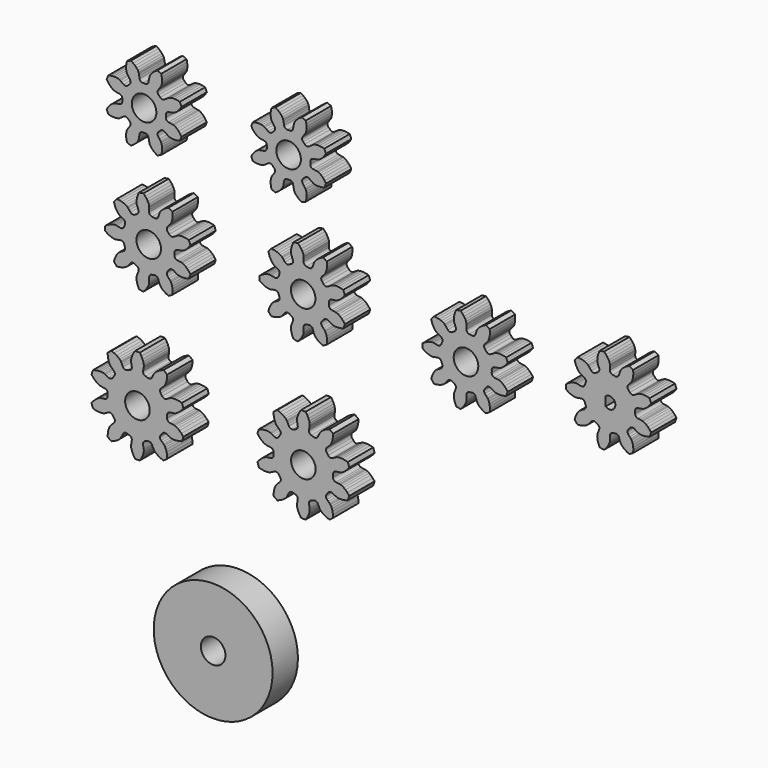
from build123d import *

# Parameters (mm, degrees)
F0_R     = 3.1
F1_DEPTH = 8
F0_R_2   = 15


# Not quite as in the source:
# - ends of sketch curves that miss each other by under 0.0002 mm in the source are joined


with BuildPart() as f1:
    # F0 (on Front) → F1 (new body)
    with BuildSketch(Plane.XZ):
        with BuildLine():
            Line((23.041986, 118.906901), (23.595075, 118.613995))
            Line((23.595075, 118.613995), (24.126006, 118.406518))
            Line((24.126006, 118.406518), (24.61132, 118.285134))
            Line((24.61132, 118.285134), (25.010692, 118.246765))
            Line((25.010692, 118.246765), (25.130189, 118.251828))
            Line((25.130189, 118.251828), (25.208747, 118.264317))
            Line((25.208747, 118.264317), (25.409385, 118.301471))
            Line((25.409385, 118.301471), (25.810146, 118.377964))
            Line((25.810146, 118.377964), (26.326841, 118.477743))
            ThreePointArc((26.326841, 118.477743), (26.9016285661, 118.3768156208), (27.2625196763, 117.9182038993))
            ThreePointArc((27.2625196763, 117.9182038993), (27.3611530691, 117.625790782), (27.4735546668, 117.3383888605))
            ThreePointArc((27.4735546668, 117.3383888605), (27.4918862395, 116.7550962402), (27.1164488836, 116.3083152097))
            Line((27.1164488836, 116.3083152097), (26.6565, 116.052626))
            Line((26.6565, 116.052626), (26.300331, 115.853618))
            Line((26.300331, 115.853618), (26.122751, 115.753112))
            Line((26.122751, 115.753112), (26.054544, 115.712183))
            Line((26.054544, 115.712183), (25.959749, 115.63925))
            Line((25.959749, 115.63925), (25.678476, 115.353147))
            Line((25.678476, 115.353147), (25.384728, 114.948207))
            Line((25.384728, 114.948207), (25.111375, 114.447994))
            Line((25.111375, 114.447994), (24.875961, 113.868097))
            Line((24.875961, 113.868097), (24.690457, 113.220615))
            ThreePointArc((24.690457, 113.220615), (25.0426662693, 112.7782581223), (25.417142014, 112.3545850131))
            Line((25.417142014, 112.3545850131), (26.086999, 112.424837))
            Line((26.086999, 112.424837), (26.698966, 112.555977))
            Line((26.698966, 112.555977), (27.239047, 112.738316))
            Line((27.239047, 112.738316), (27.688844, 112.957284))
            Line((27.688844, 112.957284), (28.019443, 113.184603))
            Line((28.019443, 113.184603), (28.107729, 113.265293))
            Line((28.107729, 113.265293), (28.15988, 113.325357))
            Line((28.15988, 113.325357), (28.289695, 113.482786))
            Line((28.289695, 113.482786), (28.547528, 113.798986))
            Line((28.547528, 113.798986), (28.879202, 114.207546))
            ThreePointArc((28.879202, 114.207546), (29.3843887373, 114.4996976362), (29.9556368617, 114.3803577848))
            ThreePointArc((29.9556368617, 114.3803577848), (30.2191551641, 114.2197567807), (30.4899990243, 114.0718440472))
            ThreePointArc((30.4899990243, 114.0718440472), (30.878974555, 113.636799028), (30.8785575696, 113.0532181649))
            Line((30.8785575696, 113.0532181649), (30.690571, 112.5617))
            Line((30.690571, 112.5617), (30.545649, 112.18031))
            Line((30.545649, 112.18031), (30.474219, 111.989172))
            Line((30.474219, 111.989172), (30.448278, 111.913977))
            Line((30.448278, 111.913977), (30.422541, 111.797173))
            Line((30.422541, 111.797173), (30.390977, 111.397207))
            Line((30.390977, 111.397207), (30.426244, 110.898188))
            Line((30.426244, 110.898188), (30.538374, 110.339294))
            Line((30.538374, 110.339294), (30.730787, 109.743745))
            Line((30.730787, 109.743745), (31.004876, 109.128506))
            ThreePointArc((31.004876, 109.128506), (31.5590253719, 109.0160366593), (32.1182219555, 108.9321926405))
            Line((32.1182219555, 108.9321926405), (32.586206, 109.416585))
            Line((32.586206, 109.416585), (32.970704, 109.910409))
            Line((32.970704, 109.910409), (33.267225, 110.397246))
            Line((33.267225, 110.397246), (33.471039, 110.854109))
            Line((33.471039, 110.854109), (33.578175, 111.24075))
            Line((33.578175, 111.24075), (33.59394, 111.359312))
            Line((33.59394, 111.359312), (33.595281, 111.438845))
            Line((33.595281, 111.438845), (33.593532, 111.642886))
            Line((33.593532, 111.642886), (33.587793, 112.050841))
            Line((33.587793, 112.050841), (33.579253, 112.577013))
            ThreePointArc((33.579253, 112.577013), (33.7784578625, 113.1255421077), (34.2927699435, 113.4013134419))
            ThreePointArc((34.2927699435, 113.4013134419), (34.5978681072, 113.447671597), (34.900422063, 113.5084587208))
            ThreePointArc((34.900422063, 113.5084587208), (35.4780365547, 113.425223725), (35.8528356986, 112.977906896))
            Line((35.8528356986, 112.977906896), (36.024772, 112.480547))
            Line((36.024772, 112.480547), (36.158908, 112.095231))
            Line((36.158908, 112.095231), (36.227051, 111.902897))
            Line((36.227051, 111.902897), (36.255514, 111.828619))
            Line((36.255514, 111.828619), (36.310878, 111.722599))
            Line((36.310878, 111.722599), (36.543792, 111.395918))
            Line((36.543792, 111.395918), (36.891571, 111.036316))
            Line((36.891571, 111.036316), (37.336717, 110.680255))
            Line((37.336717, 110.680255), (37.866925, 110.347718))
            Line((37.866925, 110.347718), (38.472358, 110.052598))
            ThreePointArc((38.472358, 110.052598), (38.9691549951, 110.3226425555), (39.451418835, 110.6178592546))
            Line((39.451418835, 110.6178592546), (39.498553, 111.289739))
            Line((39.498553, 111.289739), (39.475673, 111.915181))
            Line((39.475673, 111.915181), (39.389888, 112.47872))
            Line((39.389888, 112.47872), (39.252353, 112.959706))
            Line((39.252353, 112.959706), (39.085896, 113.324757))
            Line((39.085896, 113.324757), (39.021762, 113.425713))
            Line((39.021762, 113.425713), (38.971667, 113.487501))
            Line((38.971667, 113.487501), (38.839172, 113.642682))
            Line((38.839172, 113.642682), (38.572547, 113.951505))
            Line((38.572547, 113.951505), (38.227788, 114.349086))
            ThreePointArc((38.227788, 114.349086), (38.0278002789, 114.8973296955), (38.2445235432, 115.4391764218))
            ThreePointArc((38.2445235432, 115.4391764218), (38.4484438612, 115.6708025143), (38.6411405952, 115.9118463082))
            ThreePointArc((38.6411405952, 115.9118463082), (39.137122372, 116.2193684283), (39.7117650831, 116.1176191385))
            Line((39.7117650831, 116.1176191385), (40.163172, 115.847138))
            Line((40.163172, 115.847138), (40.513602, 115.63819))
            Line((40.513602, 115.63819), (40.689433, 115.534655))
            Line((40.689433, 115.534655), (40.758981, 115.49605))
            Line((40.758981, 115.49605), (40.86954, 115.450422))
            Line((40.86954, 115.450422), (41.25795, 115.349884))
            Line((41.25795, 115.349884), (41.755512, 115.297961))
            Line((41.755512, 115.297961), (42.325385, 115.311336))
            Line((42.325385, 115.311336), (42.945299, 115.39741))
            Line((42.945299, 115.39741), (43.598786, 115.5605))
            ThreePointArc((43.598786, 115.5605), (43.805773853, 116.0867004905), (43.9854475381, 116.6228421417))
            Line((43.9854475381, 116.6228421417), (43.589679, 117.16783))
            Line((43.589679, 117.16783), (43.170125, 117.632239))
            Line((43.170125, 117.632239), (42.742174, 118.008793))
            Line((42.742174, 118.008793), (42.327644, 118.288844))
            Line((42.327644, 118.288844), (41.965481, 118.461493))
            Line((41.965481, 118.461493), (41.851458, 118.497606))
            Line((41.851458, 118.497606), (41.773366, 118.512738))
            Line((41.773366, 118.512738), (41.572121, 118.546447))
            Line((41.572121, 118.546447), (41.169367, 118.611635))
            Line((41.169367, 118.611635), (40.649706, 118.694594))
            ThreePointArc((40.649706, 118.694594), (40.1441016582, 118.986023344), (39.9618289779, 119.540409001))
            ThreePointArc((39.9618289779, 119.540409001), (39.969155, 119.848922), (39.9618293141, 120.1574349674))
            ThreePointArc((39.9618293141, 120.1574349674), (40.1441016582, 120.711820656), (40.6497060099, 121.0032499379))
            Line((40.6497060099, 121.0032499379), (41.169367, 121.086209))
            Line((41.169367, 121.086209), (41.572121, 121.151397))
            Line((41.572121, 121.151397), (41.773366, 121.185106))
            Line((41.773366, 121.185106), (41.851458, 121.200238))
            Line((41.851458, 121.200238), (41.965481, 121.236351))
            Line((41.965481, 121.236351), (42.327644, 121.409))
            Line((42.327644, 121.409), (42.742174, 121.689051))
            Line((42.742174, 121.689051), (43.170125, 122.065605))
            Line((43.170125, 122.065605), (43.589679, 122.530014))
            Line((43.589679, 122.530014), (43.985448, 123.075002))
            ThreePointArc((43.985448, 123.075002), (43.805773853, 123.6111435095), (43.5987866775, 124.1373438635))
            Line((43.5987866775, 124.1373438635), (42.945299, 124.300434))
            Line((42.945299, 124.300434), (42.325385, 124.386508))
            Line((42.325385, 124.386508), (41.755512, 124.399883))
            Line((41.755512, 124.399883), (41.25795, 124.34796))
            Line((41.25795, 124.34796), (40.86954, 124.247422))
            Line((40.86954, 124.247422), (40.758981, 124.201794))
            Line((40.758981, 124.201794), (40.689433, 124.163189))
            Line((40.689433, 124.163189), (40.513602, 124.059654))
            Line((40.513602, 124.059654), (40.163172, 123.850706))
            Line((40.163172, 123.850706), (39.711764, 123.580225))
            ThreePointArc((39.711764, 123.580225), (39.1371221193, 123.4784756203), (38.6411405928, 123.78599669))
            ThreePointArc((38.6411405928, 123.78599669), (38.4484440973, 124.0270412043), (38.2445239971, 124.2586669973))
            ThreePointArc((38.2445239971, 124.2586669973), (38.0278002845, 124.8005139372), (38.2277886199, 125.34875833))
            Line((38.2277886199, 125.34875833), (38.572547, 125.746339))
            Line((38.572547, 125.746339), (38.839172, 126.055162))
            Line((38.839172, 126.055162), (38.971667, 126.210343))
            Line((38.971667, 126.210343), (39.021762, 126.272131))
            Line((39.021762, 126.272131), (39.085896, 126.373087))
            Line((39.085896, 126.373087), (39.252353, 126.738138))
            Line((39.252353, 126.738138), (39.389888, 127.219124))
            Line((39.389888, 127.219124), (39.475673, 127.782663))
            Line((39.475673, 127.782663), (39.498553, 128.408105))
            Line((39.498553, 128.408105), (39.451419, 129.079985))
            ThreePointArc((39.451419, 129.079985), (38.9691549951, 129.3752014445), (38.4723579137, 129.6452458311))
            Line((38.4723579137, 129.6452458311), (37.866925, 129.350126))
            Line((37.866925, 129.350126), (37.336717, 129.017589))
            Line((37.336717, 129.017589), (36.891571, 128.661528))
            Line((36.891571, 128.661528), (36.543792, 128.301926))
            Line((36.543792, 128.301926), (36.310878, 127.975245))
            Line((36.310878, 127.975245), (36.255514, 127.869225))
            Line((36.255514, 127.869225), (36.227051, 127.794947))
            Line((36.227051, 127.794947), (36.158908, 127.602613))
            Line((36.158908, 127.602613), (36.024772, 127.217297))
            Line((36.024772, 127.217297), (35.852836, 126.719937))
            ThreePointArc((35.852836, 126.719937), (35.4780365547, 126.272620275), (34.9004219689, 126.1893848621))
            ThreePointArc((34.9004219689, 126.1893848621), (34.5978681072, 126.250172403), (34.292769966, 126.2965307341))
            ThreePointArc((34.292769966, 126.2965307341), (33.778457904, 126.5723018444), (33.5792530332, 127.1208309994))
            Line((33.5792530332, 127.1208309994), (33.587793, 127.647003))
            Line((33.587793, 127.647003), (33.593532, 128.054958))
            Line((33.593532, 128.054958), (33.595281, 128.258999))
            Line((33.595281, 128.258999), (33.59394, 128.338532))
            Line((33.59394, 128.338532), (33.578175, 128.457094))
            Line((33.578175, 128.457094), (33.471039, 128.843735))
            Line((33.471039, 128.843735), (33.267225, 129.300598))
            Line((33.267225, 129.300598), (32.970704, 129.787435))
            Line((32.970704, 129.787435), (32.586206, 130.281259))
            Line((32.586206, 130.281259), (32.118222, 130.765651))
            ThreePointArc((32.118222, 130.765651), (31.5590252616, 130.6818073212), (31.0048759002, 130.569338434))
            Line((31.0048759002, 130.569338434), (30.730787, 129.954099))
            Line((30.730787, 129.954099), (30.538374, 129.35855))
            Line((30.538374, 129.35855), (30.426244, 128.799656))
            Line((30.426244, 128.799656), (30.390977, 128.300637))
            Line((30.390977, 128.300637), (30.422541, 127.900671))
            Line((30.422541, 127.900671), (30.448278, 127.783867))
            Line((30.448278, 127.783867), (30.474219, 127.708672))
            Line((30.474219, 127.708672), (30.545649, 127.517534))
            Line((30.545649, 127.517534), (30.690571, 127.136144))
            Line((30.690571, 127.136144), (30.878557, 126.644626))
            ThreePointArc((30.878557, 126.644626), (30.878974555, 126.061044972), (30.4899987994, 125.6259993889))
            ThreePointArc((30.4899987994, 125.6259993889), (30.2191549656, 125.4780871047), (29.9556370399, 125.317485938))
            ThreePointArc((29.9556370399, 125.317485938), (29.3843887373, 125.1981463638), (28.879201624, 125.4902976951))
            Line((28.879201624, 125.4902976951), (28.547528, 125.898858))
            Line((28.547528, 125.898858), (28.289695, 126.215058))
            Line((28.289695, 126.215058), (28.15988, 126.372487))
            Line((28.15988, 126.372487), (28.107729, 126.432551))
            Line((28.107729, 126.432551), (28.019443, 126.513241))
            Line((28.019443, 126.513241), (27.688844, 126.74056))
            Line((27.688844, 126.74056), (27.239047, 126.959528))
            Line((27.239047, 126.959528), (26.698966, 127.141867))
            Line((26.698966, 127.141867), (26.086999, 127.273007))
            Line((26.086999, 127.273007), (25.417142, 127.343259))
            ThreePointArc((25.417142, 127.343259), (25.0426662693, 126.9195858777), (24.6904567193, 126.477229212))
            Line((24.6904567193, 126.477229212), (24.875961, 125.829747))
            Line((24.875961, 125.829747), (25.111375, 125.24985))
            Line((25.111375, 125.24985), (25.384728, 124.749637))
            Line((25.384728, 124.749637), (25.678476, 124.344697))
            Line((25.678476, 124.344697), (25.959749, 124.058594))
            Line((25.959749, 124.058594), (26.054544, 123.985661))
            Line((26.054544, 123.985661), (26.122751, 123.944732))
            Line((26.122751, 123.944732), (26.300331, 123.844226))
            Line((26.300331, 123.844226), (26.6565, 123.645218))
            Line((26.6565, 123.645218), (27.116448, 123.389529))
            ThreePointArc((27.116448, 123.389529), (27.4918862395, 122.9427477598), (27.4735550433, 122.3594549819))
            ThreePointArc((27.4735550433, 122.3594549819), (27.3611530691, 122.072053218), (27.2625192669, 121.7796402281))
            ThreePointArc((27.2625192669, 121.7796402281), (26.9016285661, 121.3210283792), (26.3268409897, 121.220100947))
            Line((26.3268409897, 121.220100947), (25.810146, 121.31988))
            Line((25.810146, 121.31988), (25.409385, 121.396373))
            Line((25.409385, 121.396373), (25.208747, 121.433527))
            Line((25.208747, 121.433527), (25.130189, 121.446016))
            Line((25.130189, 121.446016), (25.010692, 121.451079))
            Line((25.010692, 121.451079), (24.61132, 121.41271))
            Line((24.61132, 121.41271), (24.126006, 121.291326))
            Line((24.126006, 121.291326), (23.595075, 121.083849))
            Line((23.595075, 121.083849), (23.041986, 120.790943))
            Line((23.041986, 120.790943), (22.483688, 120.414183))
            ThreePointArc((22.483688, 120.414183), (22.469155, 119.848922), (22.483688239, 119.2836609608))
            Line((22.483688239, 119.2836609608), (23.041986, 118.906901))
        make_face()
        with Locations((33.469155, 119.848922)):
            Circle(F0_R, mode=Mode.SUBTRACT)
    extrude(amount=F1_DEPTH)


with BuildPart() as f1b:
    # F0 (on Front) → F1, piece 2 (new body)
    with BuildSketch(Plane.XZ):
        with BuildLine():
            ThreePointArc((-5.3944879668, 110.9609140006), (-5.1952831375, 111.5094431077), (-4.6809710565, 111.7852144419))
            ThreePointArc((-4.6809710565, 111.7852144419), (-4.3758728928, 111.831572597), (-4.073318937, 111.8923597208))
            ThreePointArc((-4.073318937, 111.8923597208), (-3.4957044453, 111.809124725), (-3.1209053014, 111.361807896))
            Line((-3.1209053014, 111.361807896), (-2.948969, 110.864448))
            Line((-2.948969, 110.864448), (-2.814833, 110.479132))
            Line((-2.814833, 110.479132), (-2.74669, 110.286798))
            Line((-2.74669, 110.286798), (-2.718227, 110.21252))
            Line((-2.718227, 110.21252), (-2.662863, 110.1065))
            Line((-2.662863, 110.1065), (-2.429949, 109.779819))
            Line((-2.429949, 109.779819), (-2.08217, 109.420217))
            Line((-2.08217, 109.420217), (-1.637024, 109.064156))
            Line((-1.637024, 109.064156), (-1.106816, 108.731619))
            Line((-1.106816, 108.731619), (-0.501383, 108.436499))
            ThreePointArc((-0.501383, 108.436499), (-0.0045860049, 108.7065435555), (0.477677835, 109.0017602546))
            Line((0.477677835, 109.0017602546), (0.524812, 109.67364))
            Line((0.524812, 109.67364), (0.501932, 110.299082))
            Line((0.501932, 110.299082), (0.416147, 110.862621))
            Line((0.416147, 110.862621), (0.278612, 111.343607))
            Line((0.278612, 111.343607), (0.112155, 111.708658))
            Line((0.112155, 111.708658), (0.048021, 111.809614))
            Line((0.048021, 111.809614), (-0.002074, 111.871402))
            Line((-0.002074, 111.871402), (-0.134569, 112.026583))
            Line((-0.134569, 112.026583), (-0.401194, 112.335406))
            Line((-0.401194, 112.335406), (-0.745953, 112.732987))
            ThreePointArc((-0.745953, 112.732987), (-0.9459407211, 113.2812306955), (-0.7292174568, 113.8230774218))
            ThreePointArc((-0.7292174568, 113.8230774218), (-0.5252969027, 114.0547037957), (-0.3326004048, 114.2957473082))
            ThreePointArc((-0.3326004048, 114.2957473082), (0.1633808219, 114.6032693226), (0.738023642, 114.5015204032))
            Line((0.738023642, 114.5015204032), (1.189431, 114.231039))
            Line((1.189431, 114.231039), (1.539861, 114.022091))
            Line((1.539861, 114.022091), (1.715692, 113.918556))
            Line((1.715692, 113.918556), (1.78524, 113.879951))
            Line((1.78524, 113.879951), (1.895799, 113.834323))
            Line((1.895799, 113.834323), (2.284209, 113.733785))
            Line((2.284209, 113.733785), (2.781771, 113.681862))
            Line((2.781771, 113.681862), (3.351644, 113.695237))
            Line((3.351644, 113.695237), (3.971558, 113.781311))
            Line((3.971558, 113.781311), (4.625045, 113.944401))
            ThreePointArc((4.625045, 113.944401), (4.832032853, 114.4706014905), (5.0117065381, 115.0067431417))
            Line((5.0117065381, 115.0067431417), (4.615938, 115.551731))
            Line((4.615938, 115.551731), (4.196384, 116.01614))
            Line((4.196384, 116.01614), (3.768433, 116.392694))
            Line((3.768433, 116.392694), (3.353903, 116.672745))
            Line((3.353903, 116.672745), (2.99174, 116.845394))
            Line((2.99174, 116.845394), (2.877717, 116.881507))
            Line((2.877717, 116.881507), (2.799625, 116.896639))
            Line((2.799625, 116.896639), (2.59838, 116.930348))
            Line((2.59838, 116.930348), (2.195626, 116.995536))
            Line((2.195626, 116.995536), (1.675965, 117.078495))
            ThreePointArc((1.675965, 117.078495), (1.1703606582, 117.369924344), (0.9880879779, 117.924310001))
            ThreePointArc((0.9880879779, 117.924310001), (0.995414, 118.232823), (0.9880883141, 118.5413359674))
            ThreePointArc((0.9880883141, 118.5413359674), (1.1703606582, 119.095721656), (1.6759650099, 119.3871509379))
            Line((1.6759650099, 119.3871509379), (2.195626, 119.47011))
            Line((2.195626, 119.47011), (2.59838, 119.535298))
            Line((2.59838, 119.535298), (2.799625, 119.569007))
            Line((2.799625, 119.569007), (2.877717, 119.584139))
            Line((2.877717, 119.584139), (2.99174, 119.620252))
            Line((2.99174, 119.620252), (3.353903, 119.792901))
            Line((3.353903, 119.792901), (3.768433, 120.072952))
            Line((3.768433, 120.072952), (4.196384, 120.449506))
            Line((4.196384, 120.449506), (4.615938, 120.913915))
            Line((4.615938, 120.913915), (5.011707, 121.458903))
            ThreePointArc((5.011707, 121.458903), (4.832032853, 121.9950445095), (4.6250456775, 122.5212448635))
            Line((4.6250456775, 122.5212448635), (3.971558, 122.684335))
            Line((3.971558, 122.684335), (3.351644, 122.770409))
            Line((3.351644, 122.770409), (2.781771, 122.783784))
            Line((2.781771, 122.783784), (2.284209, 122.731861))
            Line((2.284209, 122.731861), (1.895799, 122.631323))
            Line((1.895799, 122.631323), (1.78524, 122.585695))
            Line((1.78524, 122.585695), (1.715692, 122.54709))
            Line((1.715692, 122.54709), (1.539861, 122.443555))
            Line((1.539861, 122.443555), (1.189431, 122.234607))
            Line((1.189431, 122.234607), (0.738023, 121.964126))
            ThreePointArc((0.738023, 121.964126), (0.1633808219, 121.8623766774), (-0.3326007741, 122.169898172))
            ThreePointArc((-0.3326007741, 122.169898172), (-0.5252971388, 122.4109424857), (-0.7292175013, 122.6425685371))
            ThreePointArc((-0.7292175013, 122.6425685371), (-0.9459407211, 123.1844153045), (-0.7459523801, 123.73265933))
            Line((-0.7459523801, 123.73265933), (-0.401194, 124.13024))
            Line((-0.401194, 124.13024), (-0.134569, 124.439063))
            Line((-0.134569, 124.439063), (-0.002074, 124.594244))
            Line((-0.002074, 124.594244), (0.048021, 124.656032))
            Line((0.048021, 124.656032), (0.112155, 124.756988))
            Line((0.112155, 124.756988), (0.278612, 125.122039))
            Line((0.278612, 125.122039), (0.416147, 125.603025))
            Line((0.416147, 125.603025), (0.501932, 126.166564))
            Line((0.501932, 126.166564), (0.524812, 126.792006))
            Line((0.524812, 126.792006), (0.477678, 127.463886))
            ThreePointArc((0.477678, 127.463886), (-0.0045860049, 127.7591024445), (-0.5013830863, 128.0291468311))
            Line((-0.5013830863, 128.0291468311), (-1.106816, 127.734027))
            Line((-1.106816, 127.734027), (-1.637024, 127.40149))
            Line((-1.637024, 127.40149), (-2.08217, 127.045429))
            Line((-2.08217, 127.045429), (-2.429949, 126.685827))
            Line((-2.429949, 126.685827), (-2.662863, 126.359146))
            Line((-2.662863, 126.359146), (-2.718227, 126.253126))
            Line((-2.718227, 126.253126), (-2.74669, 126.178848))
            Line((-2.74669, 126.178848), (-2.814833, 125.986514))
            Line((-2.814833, 125.986514), (-2.948969, 125.601198))
            Line((-2.948969, 125.601198), (-3.120905, 125.103838))
            ThreePointArc((-3.120905, 125.103838), (-3.4957044453, 124.656521275), (-4.0733190311, 124.5732858621))
            ThreePointArc((-4.0733190311, 124.5732858621), (-4.3758728928, 124.634073403), (-4.680971034, 124.6804317341))
            ThreePointArc((-4.680971034, 124.6804317341), (-5.1952831375, 124.9562028923), (-5.3944879668, 125.5047319994))
            Line((-5.3944879668, 125.5047319994), (-5.385948, 126.030904))
            Line((-5.385948, 126.030904), (-5.380209, 126.438859))
            Line((-5.380209, 126.438859), (-5.37846, 126.6429))
            Line((-5.37846, 126.6429), (-5.379801, 126.722433))
            Line((-5.379801, 126.722433), (-5.395566, 126.840995))
            Line((-5.395566, 126.840995), (-5.502702, 127.227636))
            Line((-5.502702, 127.227636), (-5.706516, 127.684499))
            Line((-5.706516, 127.684499), (-6.003037, 128.171336))
            Line((-6.003037, 128.171336), (-6.387535, 128.66516))
            Line((-6.387535, 128.66516), (-6.855519, 129.149552))
            ThreePointArc((-6.855519, 129.149552), (-7.4147157384, 129.0657083212), (-7.9688650998, 128.953239434))
            Line((-7.9688650998, 128.953239434), (-8.242954, 128.338))
            Line((-8.242954, 128.338), (-8.435367, 127.742451))
            Line((-8.435367, 127.742451), (-8.547497, 127.183557))
            Line((-8.547497, 127.183557), (-8.582764, 126.684538))
            Line((-8.582764, 126.684538), (-8.5512, 126.284572))
            Line((-8.5512, 126.284572), (-8.525463, 126.167768))
            Line((-8.525463, 126.167768), (-8.499522, 126.092573))
            Line((-8.499522, 126.092573), (-8.428092, 125.901435))
            Line((-8.428092, 125.901435), (-8.28317, 125.520045))
            Line((-8.28317, 125.520045), (-8.095184, 125.028527))
            ThreePointArc((-8.095184, 125.028527), (-8.094766445, 124.444945972), (-8.4837422006, 124.0099003889))
            ThreePointArc((-8.4837422006, 124.0099003889), (-8.7545858359, 123.8619882193), (-9.0181039601, 123.701386938))
            ThreePointArc((-9.0181039601, 123.701386938), (-9.5893522627, 123.5820473638), (-10.094539376, 123.8741986951))
            Line((-10.094539376, 123.8741986951), (-10.426213, 124.282759))
            Line((-10.426213, 124.282759), (-10.684046, 124.598959))
            Line((-10.684046, 124.598959), (-10.813861, 124.756388))
            Line((-10.813861, 124.756388), (-10.866012, 124.816452))
            Line((-10.866012, 124.816452), (-10.954298, 124.897142))
            Line((-10.954298, 124.897142), (-11.284897, 125.124461))
            Line((-11.284897, 125.124461), (-11.734694, 125.343429))
            Line((-11.734694, 125.343429), (-12.274775, 125.525768))
            Line((-12.274775, 125.525768), (-12.886742, 125.656908))
            Line((-12.886742, 125.656908), (-13.556599, 125.72716))
            ThreePointArc((-13.556599, 125.72716), (-13.9310747307, 125.3034868777), (-14.2832842807, 124.861130212))
            Line((-14.2832842807, 124.861130212), (-14.09778, 124.213648))
            Line((-14.09778, 124.213648), (-13.862366, 123.633751))
            Line((-13.862366, 123.633751), (-13.589013, 123.133538))
            Line((-13.589013, 123.133538), (-13.295265, 122.728598))
            Line((-13.295265, 122.728598), (-13.013992, 122.442495))
            Line((-13.013992, 122.442495), (-12.919197, 122.369562))
            Line((-12.919197, 122.369562), (-12.85099, 122.328633))
            Line((-12.85099, 122.328633), (-12.67341, 122.228127))
            Line((-12.67341, 122.228127), (-12.317241, 122.029119))
            Line((-12.317241, 122.029119), (-11.857293, 121.77343))
            ThreePointArc((-11.857293, 121.77343), (-11.4818549037, 121.3266491728), (-11.5001859567, 120.7433559819))
            ThreePointArc((-11.5001859567, 120.7433559819), (-11.6125879817, 120.4559540785), (-11.7112218214, 120.1635409444))
            ThreePointArc((-11.7112218214, 120.1635409444), (-12.0721124339, 119.7049293792), (-12.6469000103, 119.604001947))
            Line((-12.6469000103, 119.604001947), (-13.163595, 119.703781))
            Line((-13.163595, 119.703781), (-13.564356, 119.780274))
            Line((-13.564356, 119.780274), (-13.764994, 119.817428))
            Line((-13.764994, 119.817428), (-13.843552, 119.829917))
            Line((-13.843552, 119.829917), (-13.963049, 119.83498))
            Line((-13.963049, 119.83498), (-14.362421, 119.796611))
            Line((-14.362421, 119.796611), (-14.847735, 119.675227))
            Line((-14.847735, 119.675227), (-15.378666, 119.46775))
            Line((-15.378666, 119.46775), (-15.931755, 119.174844))
            Line((-15.931755, 119.174844), (-16.490053, 118.798084))
            ThreePointArc((-16.490053, 118.798084), (-16.504586, 118.232823), (-16.490052761, 117.6675619608))
            Line((-16.490052761, 117.6675619608), (-15.931755, 117.290802))
            Line((-15.931755, 117.290802), (-15.378666, 116.997896))
            Line((-15.378666, 116.997896), (-14.847735, 116.790419))
            Line((-14.847735, 116.790419), (-14.362421, 116.669035))
            Line((-14.362421, 116.669035), (-13.963049, 116.630666))
            Line((-13.963049, 116.630666), (-13.843552, 116.635729))
            Line((-13.843552, 116.635729), (-13.764994, 116.648218))
            Line((-13.764994, 116.648218), (-13.564356, 116.685372))
            Line((-13.564356, 116.685372), (-13.163595, 116.761865))
            Line((-13.163595, 116.761865), (-12.6469, 116.861644))
            ThreePointArc((-12.6469, 116.861644), (-12.0721124339, 116.7607166208), (-11.7112213237, 116.3021048993))
            ThreePointArc((-11.7112213237, 116.3021048993), (-11.6125879817, 116.0096919215), (-11.5001863332, 115.7222898605))
            ThreePointArc((-11.5001863332, 115.7222898605), (-11.4818549037, 115.1389968272), (-11.8572928808, 114.6922157854))
            Line((-11.8572928808, 114.6922157854), (-12.317241, 114.436527))
            Line((-12.317241, 114.436527), (-12.67341, 114.237519))
            Line((-12.67341, 114.237519), (-12.85099, 114.137013))
            Line((-12.85099, 114.137013), (-12.919197, 114.096084))
            Line((-12.919197, 114.096084), (-13.013992, 114.023151))
            Line((-13.013992, 114.023151), (-13.295265, 113.737048))
            Line((-13.295265, 113.737048), (-13.589013, 113.332108))
            Line((-13.589013, 113.332108), (-13.862366, 112.831895))
            Line((-13.862366, 112.831895), (-14.09778, 112.251998))
            Line((-14.09778, 112.251998), (-14.283284, 111.604516))
            ThreePointArc((-14.283284, 111.604516), (-13.9310747307, 111.1621591223), (-13.556598986, 110.7384860131))
            Line((-13.556598986, 110.7384860131), (-12.886742, 110.808738))
            Line((-12.886742, 110.808738), (-12.274775, 110.939878))
            Line((-12.274775, 110.939878), (-11.734694, 111.122217))
            Line((-11.734694, 111.122217), (-11.284897, 111.341185))
            Line((-11.284897, 111.341185), (-10.954298, 111.568504))
            Line((-10.954298, 111.568504), (-10.866012, 111.649194))
            Line((-10.866012, 111.649194), (-10.813861, 111.709258))
            Line((-10.813861, 111.709258), (-10.684046, 111.866687))
            Line((-10.684046, 111.866687), (-10.426213, 112.182887))
            Line((-10.426213, 112.182887), (-10.094539, 112.591447))
            ThreePointArc((-10.094539, 112.591447), (-9.5893522627, 112.8835986362), (-9.0181041383, 112.7642587848))
            ThreePointArc((-9.0181041383, 112.7642587848), (-8.7545860344, 112.6036578953), (-8.483742383, 112.4557452573))
            ThreePointArc((-8.483742383, 112.4557452573), (-8.094766445, 112.020700028), (-8.0951834304, 111.4371191649))
            Line((-8.0951834304, 111.4371191649), (-8.28317, 110.945601))
            Line((-8.28317, 110.945601), (-8.428092, 110.564211))
            Line((-8.428092, 110.564211), (-8.499522, 110.373073))
            Line((-8.499522, 110.373073), (-8.525463, 110.297878))
            Line((-8.525463, 110.297878), (-8.5512, 110.181074))
            Line((-8.5512, 110.181074), (-8.582764, 109.781108))
            Line((-8.582764, 109.781108), (-8.547497, 109.282089))
            Line((-8.547497, 109.282089), (-8.435367, 108.723195))
            Line((-8.435367, 108.723195), (-8.242954, 108.127646))
            Line((-8.242954, 108.127646), (-7.968865, 107.512407))
            ThreePointArc((-7.968865, 107.512407), (-7.4147157384, 107.3999376788), (-6.8555190445, 107.3160936405))
            Line((-6.8555190445, 107.3160936405), (-6.387535, 107.800486))
            Line((-6.387535, 107.800486), (-6.003037, 108.29431))
            Line((-6.003037, 108.29431), (-5.706516, 108.781147))
            Line((-5.706516, 108.781147), (-5.502702, 109.23801))
            Line((-5.502702, 109.23801), (-5.395566, 109.624651))
            Line((-5.395566, 109.624651), (-5.379801, 109.743213))
            Line((-5.379801, 109.743213), (-5.37846, 109.822746))
            Line((-5.37846, 109.822746), (-5.380209, 110.026787))
            Line((-5.380209, 110.026787), (-5.385948, 110.434742))
            Line((-5.385948, 110.434742), (-5.3944879668, 110.9609140006))
        make_face()
        with Locations((-5.504586, 118.232823)):
            Circle(F0_R, mode=Mode.SUBTRACT)
    extrude(amount=F1_DEPTH)


with BuildPart() as f1c:
    # F0 (on Front) → F1, piece 3 (new body)
    with BuildSketch(Plane.XZ):
        with BuildLine():
            ThreePointArc((-3.1262723189, 143.0186877791), (-3.2641737409, 143.5709303604), (-3.0026342345, 144.0764852608))
            ThreePointArc((-3.0026342345, 144.0764852608), (-2.7908177035, 144.2773467035), (-2.5899563265, 144.4891632936))
            ThreePointArc((-2.5899563265, 144.4891632936), (-2.0844013604, 144.7507027409), (-1.5321587791, 144.6128013189))
            Line((-1.5321587791, 144.6128013189), (-1.064535, 144.289254))
            Line((-1.064535, 144.289254), (-0.703867, 144.040786))
            Line((-0.703867, 144.040786), (-0.527525, 143.9207))
            Line((-0.527525, 143.9207), (-0.464027, 143.880112))
            Line((-0.464027, 143.880112), (-0.415933, 143.855271))
            Line((-0.415933, 143.855271), (-0.354979, 143.82768))
            Line((-0.354979, 143.82768), (0.024344, 143.709564))
            Line((0.024344, 143.709564), (0.51342, 143.638289))
            Line((0.51342, 143.638289), (1.076258, 143.632297))
            Line((1.076258, 143.632297), (1.69036, 143.700019))
            Line((1.69036, 143.700019), (2.338785, 143.846338))
            ThreePointArc((2.338785, 143.846338), (2.5588902651, 144.3395995316), (2.7520409875, 144.8440260044))
            Line((2.7520409875, 144.8440260044), (2.396998, 145.405995))
            Line((2.396998, 145.405995), (2.010649, 145.888118))
            Line((2.010649, 145.888118), (1.608426, 146.281867))
            Line((1.608426, 146.281867), (1.212198, 146.577297))
            Line((1.212198, 146.577297), (0.860456, 146.761999))
            Line((0.860456, 146.761999), (0.797844, 146.785589))
            Line((0.797844, 146.785589), (0.746272, 146.802032))
            Line((0.746272, 146.802032), (0.672672, 146.818231))
            Line((0.672672, 146.818231), (0.463066, 146.858011))
            Line((0.463066, 146.858011), (0.032342, 146.937348))
            Line((0.032342, 146.937348), (-0.527101, 147.039225))
            ThreePointArc((-0.527101, 147.039225), (-1.0151065708, 147.3322090589), (-1.1876513145, 147.8746270167))
            ThreePointArc((-1.1876513145, 147.8746270167), (-1.179905, 148.166434), (-1.1876514835, 148.4582409743))
            ThreePointArc((-1.1876514835, 148.4582409743), (-1.0151066262, 149.000658871), (-0.5271011019, 149.2936425609))
            Line((-0.5271011019, 149.2936425609), (0.032342, 149.39552))
            Line((0.032342, 149.39552), (0.463066, 149.474857))
            Line((0.463066, 149.474857), (0.672672, 149.514637))
            Line((0.672672, 149.514637), (0.746272, 149.530836))
            Line((0.746272, 149.530836), (0.797844, 149.547279))
            Line((0.797844, 149.547279), (0.860456, 149.570869))
            Line((0.860456, 149.570869), (1.212198, 149.755571))
            Line((1.212198, 149.755571), (1.608426, 150.051001))
            Line((1.608426, 150.051001), (2.010649, 150.44475))
            Line((2.010649, 150.44475), (2.396998, 150.926873))
            Line((2.396998, 150.926873), (2.752041, 151.488842))
            ThreePointArc((2.752041, 151.488842), (2.5588902651, 151.9932684684), (2.3387850557, 152.4865300267))
            Line((2.3387850557, 152.4865300267), (1.69036, 152.632849))
            Line((1.69036, 152.632849), (1.076258, 152.700571))
            Line((1.076258, 152.700571), (0.51342, 152.694579))
            Line((0.51342, 152.694579), (0.024344, 152.623304))
            Line((0.024344, 152.623304), (-0.354979, 152.505188))
            Line((-0.354979, 152.505188), (-0.415933, 152.477597))
            Line((-0.415933, 152.477597), (-0.464027, 152.452756))
            Line((-0.464027, 152.452756), (-0.527525, 152.412168))
            Line((-0.527525, 152.412168), (-0.703867, 152.292082))
            Line((-0.703867, 152.292082), (-1.064535, 152.043614))
            Line((-1.064535, 152.043614), (-1.532159, 151.720066))
            ThreePointArc((-1.532159, 151.720066), (-2.0844012739, 151.582165249), (-2.5899557636, 151.8437042125))
            ThreePointArc((-2.5899557636, 151.8437042125), (-2.7908172042, 152.0555207972), (-3.0026337964, 152.2563822265))
            ThreePointArc((-3.0026337964, 152.2563822265), (-3.2641736543, 152.7619368993), (-3.126272787, 153.3141795451))
            Line((-3.126272787, 153.3141795451), (-2.802725, 153.781804))
            Line((-2.802725, 153.781804), (-2.554257, 154.142472))
            Line((-2.554257, 154.142472), (-2.434171, 154.318814))
            Line((-2.434171, 154.318814), (-2.393583, 154.382312))
            Line((-2.393583, 154.382312), (-2.368742, 154.430406))
            Line((-2.368742, 154.430406), (-2.341151, 154.49136))
            Line((-2.341151, 154.49136), (-2.223035, 154.870683))
            Line((-2.223035, 154.870683), (-2.15176, 155.359759))
            Line((-2.15176, 155.359759), (-2.145768, 155.922597))
            Line((-2.145768, 155.922597), (-2.21349, 156.536699))
            Line((-2.21349, 156.536699), (-2.359809, 157.185124))
            ThreePointArc((-2.359809, 157.185124), (-2.8530705316, 157.4052292651), (-3.3574970044, 157.5983799875))
            Line((-3.3574970044, 157.5983799875), (-3.919466, 157.243337))
            Line((-3.919466, 157.243337), (-4.401589, 156.856988))
            Line((-4.401589, 156.856988), (-4.795338, 156.454765))
            Line((-4.795338, 156.454765), (-5.090768, 156.058537))
            Line((-5.090768, 156.058537), (-5.27547, 155.706795))
            Line((-5.27547, 155.706795), (-5.29906, 155.644183))
            Line((-5.29906, 155.644183), (-5.315503, 155.592611))
            Line((-5.315503, 155.592611), (-5.331702, 155.519011))
            Line((-5.331702, 155.519011), (-5.371482, 155.309405))
            Line((-5.371482, 155.309405), (-5.450819, 154.878681))
            Line((-5.450819, 154.878681), (-5.552696, 154.319238))
            ThreePointArc((-5.552696, 154.319238), (-5.8456800381, 153.8312324457), (-6.3880979637, 153.6586876827))
            ThreePointArc((-6.3880979637, 153.6586876827), (-6.679905, 153.666434), (-6.9717120273, 153.6586875137))
            ThreePointArc((-6.9717120273, 153.6586875137), (-7.5141298918, 153.8312323903), (-7.8071135609, 154.3192378981))
            Line((-7.8071135609, 154.3192378981), (-7.908991, 154.878681))
            Line((-7.908991, 154.878681), (-7.988328, 155.309405))
            Line((-7.988328, 155.309405), (-8.028108, 155.519011))
            Line((-8.028108, 155.519011), (-8.044307, 155.592611))
            Line((-8.044307, 155.592611), (-8.06075, 155.644183))
            Line((-8.06075, 155.644183), (-8.08434, 155.706795))
            Line((-8.08434, 155.706795), (-8.269042, 156.058537))
            Line((-8.269042, 156.058537), (-8.564472, 156.454765))
            Line((-8.564472, 156.454765), (-8.958221, 156.856988))
            Line((-8.958221, 156.856988), (-9.440344, 157.243337))
            Line((-9.440344, 157.243337), (-10.002313, 157.59838))
            ThreePointArc((-10.002313, 157.59838), (-10.5067394684, 157.4052292651), (-11.0000010267, 157.1851240557))
            Line((-11.0000010267, 157.1851240557), (-11.14632, 156.536699))
            Line((-11.14632, 156.536699), (-11.214042, 155.922597))
            Line((-11.214042, 155.922597), (-11.20805, 155.359759))
            Line((-11.20805, 155.359759), (-11.136775, 154.870683))
            Line((-11.136775, 154.870683), (-11.018659, 154.49136))
            Line((-11.018659, 154.49136), (-10.991068, 154.430406))
            Line((-10.991068, 154.430406), (-10.966227, 154.382312))
            Line((-10.966227, 154.382312), (-10.925639, 154.318814))
            Line((-10.925639, 154.318814), (-10.805553, 154.142472))
            Line((-10.805553, 154.142472), (-10.557085, 153.781804))
            Line((-10.557085, 153.781804), (-10.233537, 153.31418))
            ThreePointArc((-10.233537, 153.31418), (-10.0956363787, 152.7619366166), (-10.3571762627, 152.2563822922))
            ThreePointArc((-10.3571762627, 152.2563822922), (-10.5689927958, 152.0555207972), (-10.7698541707, 151.8437041534))
            ThreePointArc((-10.7698541707, 151.8437041534), (-11.2754087261, 151.582165249), (-11.8276507528, 151.7200663569))
            Line((-11.8276507528, 151.7200663569), (-12.295275, 152.043614))
            Line((-12.295275, 152.043614), (-12.655943, 152.292082))
            Line((-12.655943, 152.292082), (-12.832285, 152.412168))
            Line((-12.832285, 152.412168), (-12.895783, 152.452756))
            Line((-12.895783, 152.452756), (-12.943877, 152.477597))
            Line((-12.943877, 152.477597), (-13.004831, 152.505188))
            Line((-13.004831, 152.505188), (-13.384154, 152.623304))
            Line((-13.384154, 152.623304), (-13.87323, 152.694579))
            Line((-13.87323, 152.694579), (-14.436068, 152.700571))
            Line((-14.436068, 152.700571), (-15.05017, 152.632849))
            Line((-15.05017, 152.632849), (-15.698595, 152.48653))
            ThreePointArc((-15.698595, 152.48653), (-15.9187002651, 151.9932684684), (-16.1118509875, 151.4888419956))
            Line((-16.1118509875, 151.4888419956), (-15.756808, 150.926873))
            Line((-15.756808, 150.926873), (-15.370459, 150.44475))
            Line((-15.370459, 150.44475), (-14.968236, 150.051001))
            Line((-14.968236, 150.051001), (-14.572008, 149.755571))
            Line((-14.572008, 149.755571), (-14.220266, 149.570869))
            Line((-14.220266, 149.570869), (-14.157654, 149.547279))
            Line((-14.157654, 149.547279), (-14.106082, 149.530836))
            Line((-14.106082, 149.530836), (-14.032482, 149.514637))
            Line((-14.032482, 149.514637), (-13.822876, 149.474857))
            Line((-13.822876, 149.474857), (-13.392152, 149.39552))
            Line((-13.392152, 149.39552), (-12.832709, 149.293643))
            ThreePointArc((-12.832709, 149.293643), (-12.3447033738, 149.000658871), (-12.1721586855, 148.4582409833))
            ThreePointArc((-12.1721586855, 148.4582409833), (-12.179905, 148.166434), (-12.1721585137, 147.8746269727))
            ThreePointArc((-12.1721585137, 147.8746269727), (-12.3447034292, 147.3322090589), (-12.8327090739, 147.0392254071))
            Line((-12.8327090739, 147.0392254071), (-13.392152, 146.937348))
            Line((-13.392152, 146.937348), (-13.822876, 146.858011))
            Line((-13.822876, 146.858011), (-14.032482, 146.818231))
            Line((-14.032482, 146.818231), (-14.106082, 146.802032))
            Line((-14.106082, 146.802032), (-14.157654, 146.785589))
            Line((-14.157654, 146.785589), (-14.220266, 146.761999))
            Line((-14.220266, 146.761999), (-14.572008, 146.577297))
            Line((-14.572008, 146.577297), (-14.968236, 146.281867))
            Line((-14.968236, 146.281867), (-15.370459, 145.888118))
            Line((-15.370459, 145.888118), (-15.756808, 145.405995))
            Line((-15.756808, 145.405995), (-16.111851, 144.844026))
            ThreePointArc((-16.111851, 144.844026), (-15.9187002651, 144.3395995316), (-15.6985950557, 143.8463379733))
            Line((-15.6985950557, 143.8463379733), (-15.05017, 143.700019))
            Line((-15.05017, 143.700019), (-14.436068, 143.632297))
            Line((-14.436068, 143.632297), (-13.87323, 143.638289))
            Line((-13.87323, 143.638289), (-13.384154, 143.709564))
            Line((-13.384154, 143.709564), (-13.004831, 143.82768))
            Line((-13.004831, 143.82768), (-12.943877, 143.855271))
            Line((-12.943877, 143.855271), (-12.895783, 143.880112))
            Line((-12.895783, 143.880112), (-12.832285, 143.9207))
            Line((-12.832285, 143.9207), (-12.655943, 144.040786))
            Line((-12.655943, 144.040786), (-12.295275, 144.289254))
            Line((-12.295275, 144.289254), (-11.827651, 144.612802))
            ThreePointArc((-11.827651, 144.612802), (-11.2754086396, 144.7507027409), (-10.7698537392, 144.4891632345))
            ThreePointArc((-10.7698537392, 144.4891632345), (-10.5689922965, 144.2773467035), (-10.3571757064, 144.0764853265))
            ThreePointArc((-10.3571757064, 144.0764853265), (-10.0956362922, 143.5709306432), (-10.2335373569, 143.0186882472))
            Line((-10.2335373569, 143.0186882472), (-10.557085, 142.551064))
            Line((-10.557085, 142.551064), (-10.805553, 142.190396))
            Line((-10.805553, 142.190396), (-10.925639, 142.014054))
            Line((-10.925639, 142.014054), (-10.966227, 141.950556))
            Line((-10.966227, 141.950556), (-10.991068, 141.902462))
            Line((-10.991068, 141.902462), (-11.018659, 141.841508))
            Line((-11.018659, 141.841508), (-11.136775, 141.462185))
            Line((-11.136775, 141.462185), (-11.20805, 140.973109))
            Line((-11.20805, 140.973109), (-11.214042, 140.410271))
            Line((-11.214042, 140.410271), (-11.14632, 139.796169))
            Line((-11.14632, 139.796169), (-11.000001, 139.147744))
            ThreePointArc((-11.000001, 139.147744), (-10.5067394684, 138.9276387349), (-10.0023129956, 138.7344880125))
            Line((-10.0023129956, 138.7344880125), (-9.440344, 139.089531))
            Line((-9.440344, 139.089531), (-8.958221, 139.47588))
            Line((-8.958221, 139.47588), (-8.564472, 139.878103))
            Line((-8.564472, 139.878103), (-8.269042, 140.274331))
            Line((-8.269042, 140.274331), (-8.08434, 140.626073))
            Line((-8.08434, 140.626073), (-8.06075, 140.688685))
            Line((-8.06075, 140.688685), (-8.044307, 140.740257))
            Line((-8.044307, 140.740257), (-8.028108, 140.813857))
            Line((-8.028108, 140.813857), (-7.988328, 141.023463))
            Line((-7.988328, 141.023463), (-7.908991, 141.454187))
            Line((-7.908991, 141.454187), (-7.807114, 142.01363))
            ThreePointArc((-7.807114, 142.01363), (-7.514129871, 142.5016356262), (-6.9717119833, 142.6741803145))
            ThreePointArc((-6.9717119833, 142.6741803145), (-6.679905, 142.666434), (-6.3880980257, 142.6741804835))
            ThreePointArc((-6.3880980257, 142.6741804835), (-5.8456800589, 142.5016355708), (-5.5526964071, 142.0136299261))
            Line((-5.5526964071, 142.0136299261), (-5.450819, 141.454187))
            Line((-5.450819, 141.454187), (-5.371482, 141.023463))
            Line((-5.371482, 141.023463), (-5.331702, 140.813857))
            Line((-5.331702, 140.813857), (-5.315503, 140.740257))
            Line((-5.315503, 140.740257), (-5.29906, 140.688685))
            Line((-5.29906, 140.688685), (-5.27547, 140.626073))
            Line((-5.27547, 140.626073), (-5.090768, 140.274331))
            Line((-5.090768, 140.274331), (-4.795338, 139.878103))
            Line((-4.795338, 139.878103), (-4.401589, 139.47588))
            Line((-4.401589, 139.47588), (-3.919466, 139.089531))
            Line((-3.919466, 139.089531), (-3.357497, 138.734488))
            ThreePointArc((-3.357497, 138.734488), (-2.8530705316, 138.9276387349), (-2.3598089733, 139.1477439443))
            Line((-2.3598089733, 139.1477439443), (-2.21349, 139.796169))
            Line((-2.21349, 139.796169), (-2.145768, 140.410271))
            Line((-2.145768, 140.410271), (-2.15176, 140.973109))
            Line((-2.15176, 140.973109), (-2.223035, 141.462185))
            Line((-2.223035, 141.462185), (-2.341151, 141.841508))
            Line((-2.341151, 141.841508), (-2.368742, 141.902462))
            Line((-2.368742, 141.902462), (-2.393583, 141.950556))
            Line((-2.393583, 141.950556), (-2.434171, 142.014054))
            Line((-2.434171, 142.014054), (-2.554257, 142.190396))
            Line((-2.554257, 142.190396), (-2.802725, 142.551064))
            Line((-2.802725, 142.551064), (-3.1262723189, 143.0186877791))
        make_face()
        with Locations((-6.679905, 148.166434)):
            Circle(F0_R, mode=Mode.SUBTRACT)
    extrude(amount=F1_DEPTH)


with BuildPart() as f1d:
    # F0 (on Front) → F1, piece 4 (new body)
    with BuildSketch(Plane.XZ):
        with BuildLine():
            Line((32.555525, 158.70128), (32.073402, 158.314931))
            Line((32.073402, 158.314931), (31.679653, 157.912708))
            Line((31.679653, 157.912708), (31.384223, 157.51648))
            Line((31.384223, 157.51648), (31.199521, 157.164738))
            Line((31.199521, 157.164738), (31.175931, 157.102126))
            Line((31.175931, 157.102126), (31.159488, 157.050554))
            Line((31.159488, 157.050554), (31.143289, 156.976954))
            Line((31.143289, 156.976954), (31.103509, 156.767348))
            Line((31.103509, 156.767348), (31.024172, 156.336624))
            Line((31.024172, 156.336624), (30.922295, 155.777181))
            ThreePointArc((30.922295, 155.777181), (30.629311327, 155.2891757343), (30.0868929833, 155.1166306855))
            ThreePointArc((30.0868929833, 155.1166306855), (29.795086, 155.124377), (29.5032790257, 155.1166305165))
            ThreePointArc((29.5032790257, 155.1166305165), (28.960860673, 155.2891757343), (28.6678772314, 155.777182042))
            Line((28.6678772314, 155.777182042), (28.566, 156.336624))
            Line((28.566, 156.336624), (28.486663, 156.767348))
            Line((28.486663, 156.767348), (28.446883, 156.976954))
            Line((28.446883, 156.976954), (28.430684, 157.050554))
            Line((28.430684, 157.050554), (28.414241, 157.102126))
            Line((28.414241, 157.102126), (28.390651, 157.164738))
            Line((28.390651, 157.164738), (28.205949, 157.51648))
            Line((28.205949, 157.51648), (27.910519, 157.912708))
            Line((27.910519, 157.912708), (27.51677, 158.314931))
            Line((27.51677, 158.314931), (27.034647, 158.70128))
            Line((27.034647, 158.70128), (26.472678, 159.056323))
            ThreePointArc((26.472678, 159.056323), (25.9682517311, 158.8631723478), (25.4749903629, 158.6430672423))
            Line((25.4749903629, 158.6430672423), (25.328671, 157.994642))
            Line((25.328671, 157.994642), (25.260949, 157.38054))
            Line((25.260949, 157.38054), (25.266941, 156.817702))
            Line((25.266941, 156.817702), (25.338216, 156.328626))
            Line((25.338216, 156.328626), (25.456332, 155.949303))
            Line((25.456332, 155.949303), (25.483923, 155.888349))
            Line((25.483923, 155.888349), (25.508764, 155.840255))
            Line((25.508764, 155.840255), (25.549352, 155.776757))
            Line((25.549352, 155.776757), (25.669438, 155.600415))
            Line((25.669438, 155.600415), (25.917906, 155.239747))
            Line((25.917906, 155.239747), (26.241454, 154.772123))
            ThreePointArc((26.241454, 154.772123), (26.3793547078, 154.2198803568), (26.1178152345, 153.7143257392))
            ThreePointArc((26.1178152345, 153.7143257392), (25.9059987035, 153.5134642965), (25.7051373265, 153.3016477064))
            ThreePointArc((25.7051373265, 153.3016477064), (25.1995823604, 153.0401082591), (24.6473397791, 153.1780096811))
            Line((24.6473397791, 153.1780096811), (24.179716, 153.501557))
            Line((24.179716, 153.501557), (23.819048, 153.750025))
            Line((23.819048, 153.750025), (23.642706, 153.870111))
            Line((23.642706, 153.870111), (23.579208, 153.910699))
            Line((23.579208, 153.910699), (23.531114, 153.93554))
            Line((23.531114, 153.93554), (23.47016, 153.963131))
            Line((23.47016, 153.963131), (23.090837, 154.081247))
            Line((23.090837, 154.081247), (22.601761, 154.152522))
            Line((22.601761, 154.152522), (22.038923, 154.158514))
            Line((22.038923, 154.158514), (21.424821, 154.090792))
            Line((21.424821, 154.090792), (20.776396, 153.944473))
            ThreePointArc((20.776396, 153.944473), (20.5562909074, 153.4512118851), (20.3631400125, 152.9467849956))
            Line((20.3631400125, 152.9467849956), (20.718183, 152.384816))
            Line((20.718183, 152.384816), (21.104532, 151.902693))
            Line((21.104532, 151.902693), (21.506755, 151.508944))
            Line((21.506755, 151.508944), (21.902983, 151.213514))
            Line((21.902983, 151.213514), (22.254725, 151.028812))
            Line((22.254725, 151.028812), (22.317337, 151.005222))
            Line((22.317337, 151.005222), (22.368909, 150.988779))
            Line((22.368909, 150.988779), (22.442509, 150.97258))
            Line((22.442509, 150.97258), (22.652115, 150.9328))
            Line((22.652115, 150.9328), (23.082839, 150.853463))
            Line((23.082839, 150.853463), (23.642282, 150.751586))
            ThreePointArc((23.642282, 150.751586), (24.1302875708, 150.4586019411), (24.3028323145, 149.9161839833))
            ThreePointArc((24.3028323145, 149.9161839833), (24.295086, 149.6243774993), (24.3028324305, 149.3325710229))
            ThreePointArc((24.3028324305, 149.3325710229), (24.1302879359, 148.7901525207), (23.6422821019, 148.4971684391))
            Line((23.6422821019, 148.4971684391), (23.082839, 148.395291))
            Line((23.082839, 148.395291), (22.652115, 148.315954))
            Line((22.652115, 148.315954), (22.442509, 148.276174))
            Line((22.442509, 148.276174), (22.368909, 148.259975))
            Line((22.368909, 148.259975), (22.317337, 148.243532))
            Line((22.317337, 148.243532), (22.254725, 148.219942))
            Line((22.254725, 148.219942), (21.902983, 148.03524))
            Line((21.902983, 148.03524), (21.506755, 147.73981))
            Line((21.506755, 147.73981), (21.104532, 147.346061))
            Line((21.104532, 147.346061), (20.718183, 146.863938))
            Line((20.718183, 146.863938), (20.36314, 146.301969))
            ThreePointArc((20.36314, 146.301969), (20.5562907349, 145.7975425316), (20.7763959443, 145.3042809733))
            Line((20.7763959443, 145.3042809733), (21.424821, 145.157962))
            Line((21.424821, 145.157962), (22.038923, 145.09024))
            Line((22.038923, 145.09024), (22.601761, 145.096232))
            Line((22.601761, 145.096232), (23.090837, 145.167507))
            Line((23.090837, 145.167507), (23.47016, 145.285623))
            Line((23.47016, 145.285623), (23.531114, 145.313214))
            Line((23.531114, 145.313214), (23.579208, 145.338055))
            Line((23.579208, 145.338055), (23.642706, 145.378643))
            Line((23.642706, 145.378643), (23.819048, 145.498729))
            Line((23.819048, 145.498729), (24.179716, 145.747197))
            Line((24.179716, 145.747197), (24.64734, 146.070745))
            ThreePointArc((24.64734, 146.070745), (25.1995822739, 146.208645751), (25.7051367636, 145.9471067875))
            ThreePointArc((25.7051367636, 145.9471067875), (25.9059982042, 145.7352902028), (26.1178147964, 145.5344287735))
            ThreePointArc((26.1178147964, 145.5344287735), (26.3793546213, 145.0288743834), (26.2414541112, 144.476631923))
            Line((26.2414541112, 144.476631923), (25.917906, 144.009007))
            Line((25.917906, 144.009007), (25.669438, 143.648339))
            Line((25.669438, 143.648339), (25.549352, 143.471997))
            Line((25.549352, 143.471997), (25.508764, 143.408499))
            Line((25.508764, 143.408499), (25.483923, 143.360405))
            Line((25.483923, 143.360405), (25.456332, 143.299451))
            Line((25.456332, 143.299451), (25.338216, 142.920128))
            Line((25.338216, 142.920128), (25.266941, 142.431052))
            Line((25.266941, 142.431052), (25.260949, 141.868214))
            Line((25.260949, 141.868214), (25.328671, 141.254112))
            Line((25.328671, 141.254112), (25.47499, 140.605687))
            ThreePointArc((25.47499, 140.605687), (25.9682513781, 140.3855817984), (26.472677691, 140.1924311229))
            Line((26.472677691, 140.1924311229), (27.034647, 140.547474))
            Line((27.034647, 140.547474), (27.51677, 140.933823))
            Line((27.51677, 140.933823), (27.910519, 141.336046))
            Line((27.910519, 141.336046), (28.205949, 141.732274))
            Line((28.205949, 141.732274), (28.390651, 142.084016))
            Line((28.390651, 142.084016), (28.414241, 142.146628))
            Line((28.414241, 142.146628), (28.430684, 142.1982))
            Line((28.430684, 142.1982), (28.446883, 142.2718))
            Line((28.446883, 142.2718), (28.486663, 142.481406))
            Line((28.486663, 142.481406), (28.566, 142.91213))
            Line((28.566, 142.91213), (28.667877, 143.471573))
            ThreePointArc((28.667877, 143.471573), (28.9608610381, 143.9595785543), (29.5032789637, 144.1321233173))
            ThreePointArc((29.5032789637, 144.1321233173), (29.795086, 144.124377), (30.0868930273, 144.1321234863))
            ThreePointArc((30.0868930273, 144.1321234863), (30.6293109619, 143.9595785543), (30.9222945929, 143.4715729261))
            Line((30.9222945929, 143.4715729261), (31.024172, 142.91213))
            Line((31.024172, 142.91213), (31.103509, 142.481406))
            Line((31.103509, 142.481406), (31.143289, 142.2718))
            Line((31.143289, 142.2718), (31.159488, 142.1982))
            Line((31.159488, 142.1982), (31.175931, 142.146628))
            Line((31.175931, 142.146628), (31.199521, 142.084016))
            Line((31.199521, 142.084016), (31.384223, 141.732274))
            Line((31.384223, 141.732274), (31.679653, 141.336046))
            Line((31.679653, 141.336046), (32.073402, 140.933823))
            Line((32.073402, 140.933823), (32.555525, 140.547474))
            Line((32.555525, 140.547474), (33.117494, 140.192431))
            ThreePointArc((33.117494, 140.192431), (33.6219206219, 140.3855817984), (34.1151820267, 140.6056869443))
            Line((34.1151820267, 140.6056869443), (34.261501, 141.254112))
            Line((34.261501, 141.254112), (34.329223, 141.868214))
            Line((34.329223, 141.868214), (34.323231, 142.431052))
            Line((34.323231, 142.431052), (34.251956, 142.920128))
            Line((34.251956, 142.920128), (34.13384, 143.299451))
            Line((34.13384, 143.299451), (34.106249, 143.360405))
            Line((34.106249, 143.360405), (34.081408, 143.408499))
            Line((34.081408, 143.408499), (34.04082, 143.471997))
            Line((34.04082, 143.471997), (33.920734, 143.648339))
            Line((33.920734, 143.648339), (33.672266, 144.009007))
            Line((33.672266, 144.009007), (33.348718, 144.476631))
            ThreePointArc((33.348718, 144.476631), (33.2108173787, 145.0288743834), (33.4723572627, 145.5344287078))
            ThreePointArc((33.4723572627, 145.5344287078), (33.6841737958, 145.7352902028), (33.8850351707, 145.9471068466))
            ThreePointArc((33.8850351707, 145.9471068466), (34.3905897261, 146.208645751), (34.9428317528, 146.0707446431))
            Line((34.9428317528, 146.0707446431), (35.410456, 145.747197))
            Line((35.410456, 145.747197), (35.771124, 145.498729))
            Line((35.771124, 145.498729), (35.947466, 145.378643))
            Line((35.947466, 145.378643), (36.010964, 145.338055))
            Line((36.010964, 145.338055), (36.059058, 145.313214))
            Line((36.059058, 145.313214), (36.120012, 145.285623))
            Line((36.120012, 145.285623), (36.499335, 145.167507))
            Line((36.499335, 145.167507), (36.988411, 145.096232))
            Line((36.988411, 145.096232), (37.551249, 145.09024))
            Line((37.551249, 145.09024), (38.165351, 145.157962))
            Line((38.165351, 145.157962), (38.813776, 145.304281))
            ThreePointArc((38.813776, 145.304281), (39.0338812651, 145.7975425316), (39.2270319875, 146.3019690044))
            Line((39.2270319875, 146.3019690044), (38.871989, 146.863938))
            Line((38.871989, 146.863938), (38.48564, 147.346061))
            Line((38.48564, 147.346061), (38.083417, 147.73981))
            Line((38.083417, 147.73981), (37.687189, 148.03524))
            Line((37.687189, 148.03524), (37.335447, 148.219942))
            Line((37.335447, 148.219942), (37.272835, 148.243532))
            Line((37.272835, 148.243532), (37.221263, 148.259975))
            Line((37.221263, 148.259975), (37.147663, 148.276174))
            Line((37.147663, 148.276174), (36.938057, 148.315954))
            Line((36.938057, 148.315954), (36.507333, 148.395291))
            Line((36.507333, 148.395291), (35.94789, 148.497168))
            ThreePointArc((35.94789, 148.497168), (35.4598840641, 148.7901525207), (35.2873397385, 149.3325710139))
            ThreePointArc((35.2873397385, 149.3325710139), (35.295086, 149.6243774993), (35.2873395165, 149.9161839743))
            ThreePointArc((35.2873395165, 149.9161839743), (35.4598844292, 150.4586019411), (35.9478900739, 150.7515855929))
            Line((35.9478900739, 150.7515855929), (36.507333, 150.853463))
            Line((36.507333, 150.853463), (36.938057, 150.9328))
            Line((36.938057, 150.9328), (37.147663, 150.97258))
            Line((37.147663, 150.97258), (37.221263, 150.988779))
            Line((37.221263, 150.988779), (37.272835, 151.005222))
            Line((37.272835, 151.005222), (37.335447, 151.028812))
            Line((37.335447, 151.028812), (37.687189, 151.213514))
            Line((37.687189, 151.213514), (38.083417, 151.508944))
            Line((38.083417, 151.508944), (38.48564, 151.902693))
            Line((38.48564, 151.902693), (38.871989, 152.384816))
            Line((38.871989, 152.384816), (39.227032, 152.946785))
            ThreePointArc((39.227032, 152.946785), (39.0338810926, 153.4512118851), (38.8137756661, 153.94447384))
            Line((38.8137756661, 153.94447384), (38.165351, 154.090792))
            Line((38.165351, 154.090792), (37.551249, 154.158514))
            Line((37.551249, 154.158514), (36.988411, 154.152522))
            Line((36.988411, 154.152522), (36.499335, 154.081247))
            Line((36.499335, 154.081247), (36.120012, 153.963131))
            Line((36.120012, 153.963131), (36.059058, 153.93554))
            Line((36.059058, 153.93554), (36.010964, 153.910699))
            Line((36.010964, 153.910699), (35.947466, 153.870111))
            Line((35.947466, 153.870111), (35.771124, 153.750025))
            Line((35.771124, 153.750025), (35.410456, 153.501557))
            Line((35.410456, 153.501557), (34.942832, 153.178009))
            ThreePointArc((34.942832, 153.178009), (34.3905896396, 153.0401082591), (33.8850347392, 153.3016477655))
            ThreePointArc((33.8850347392, 153.3016477655), (33.6841732965, 153.5134642965), (33.4723567064, 153.7143256735))
            ThreePointArc((33.4723567064, 153.7143256735), (33.2108172922, 154.2198803568), (33.3487183569, 154.7721227528))
            Line((33.3487183569, 154.7721227528), (33.672266, 155.239747))
            Line((33.672266, 155.239747), (33.920734, 155.600415))
            Line((33.920734, 155.600415), (34.04082, 155.776757))
            Line((34.04082, 155.776757), (34.081408, 155.840255))
            Line((34.081408, 155.840255), (34.106249, 155.888349))
            Line((34.106249, 155.888349), (34.13384, 155.949303))
            Line((34.13384, 155.949303), (34.251956, 156.328626))
            Line((34.251956, 156.328626), (34.323231, 156.817702))
            Line((34.323231, 156.817702), (34.329223, 157.38054))
            Line((34.329223, 157.38054), (34.261501, 157.994642))
            Line((34.261501, 157.994642), (34.115182, 158.643067))
            ThreePointArc((34.115182, 158.643067), (33.6219202689, 158.8631723478), (33.1174939956, 159.0563229875))
            Line((33.1174939956, 159.0563229875), (32.555525, 158.70128))
        make_face()
        with Locations((29.795086, 149.624377)):
            Circle(F0_R, mode=Mode.SUBTRACT)
    extrude(amount=F1_DEPTH)


with BuildPart() as f1e:
    # F0 (on Front) → F1, piece 5 (new body)
    with BuildSketch(Plane.XZ):
        with BuildLine():
            Line((-6.786559, 90.49591), (-6.754115, 90.689813))
            Line((-6.754115, 90.689813), (-6.741392, 90.776516))
            Line((-6.741392, 90.776516), (-6.73729, 90.891415))
            Line((-6.73729, 90.891415), (-6.771291, 91.264281))
            Line((-6.771291, 91.264281), (-6.876317, 91.718887))
            Line((-6.876317, 91.718887), (-7.055293, 92.219167))
            Line((-7.055293, 92.219167), (-7.360851, 92.840099))
            Line((-7.360851, 92.840099), (-7.766648, 93.473062))
            ThreePointArc((-7.766648, 93.473062), (-8.353491, 93.48742), (-8.9403340023, 93.4730620475))
            Line((-8.9403340023, 93.4730620475), (-9.346131, 92.840099))
            Line((-9.346131, 92.840099), (-9.651689, 92.219167))
            Line((-9.651689, 92.219167), (-9.830665, 91.718887))
            Line((-9.830665, 91.718887), (-9.935691, 91.264281))
            Line((-9.935691, 91.264281), (-9.969692, 90.891415))
            Line((-9.969692, 90.891415), (-9.96559, 90.776516))
            Line((-9.96559, 90.776516), (-9.952867, 90.689813))
            Line((-9.952867, 90.689813), (-9.920423, 90.49591))
            Line((-9.920423, 90.49591), (-9.856065, 90.123417))
            Line((-9.856065, 90.123417), (-9.773016, 89.649051))
            ThreePointArc((-9.773016, 89.649051), (-9.8876164858, 89.0671121103), (-10.3634721568, 88.7130675638))
            ThreePointArc((-10.3634721568, 88.7130675638), (-10.6711185445, 88.6203438441), (-10.9745111704, 88.514528457))
            ThreePointArc((-10.9745111704, 88.514528457), (-11.5675889938, 88.5212563918), (-12.0023574015, 88.9246942924))
            Line((-12.0023574015, 88.9246942924), (-12.213994, 89.357279))
            Line((-12.213994, 89.357279), (-12.380874, 89.696461))
            Line((-12.380874, 89.696461), (-12.468599, 89.872402))
            Line((-12.468599, 89.872402), (-12.509269, 89.950025))
            Line((-12.509269, 89.950025), (-12.573487, 90.045391))
            Line((-12.573487, 90.045391), (-12.820159, 90.32706))
            Line((-12.820159, 90.32706), (-13.172338, 90.633112))
            Line((-13.172338, 90.633112), (-13.61119, 90.932647))
            Line((-13.61119, 90.932647), (-14.223365, 91.255389))
            Line((-14.223365, 91.255389), (-14.923709, 91.528946))
            ThreePointArc((-14.923709, 91.528946), (-15.4069137573, 91.1956241288), (-15.8732399622, 90.839070953))
            Line((-15.8732399622, 90.839070953), (-15.829491, 90.088471))
            Line((-15.829491, 90.088471), (-15.711718, 89.406524))
            Line((-15.711718, 89.406524), (-15.562455, 88.89659))
            Line((-15.562455, 88.89659), (-15.380212, 88.467073))
            Line((-15.380212, 88.467073), (-15.188554, 88.145433))
            Line((-15.188554, 88.145433), (-15.1177, 88.054889))
            Line((-15.1177, 88.054889), (-15.056445, 87.992223))
            Line((-15.056445, 87.992223), (-14.916224, 87.854422))
            Line((-14.916224, 87.854422), (-14.645211, 87.590897))
            Line((-14.645211, 87.590897), (-14.299197, 87.255943))
            ThreePointArc((-14.299197, 87.255943), (-14.0498557405, 86.7177834057), (-14.2267290969, 86.151654077))
            ThreePointArc((-14.2267290969, 86.151654077), (-14.4211187116, 85.895809043), (-14.6043717808, 85.6318728547))
            ThreePointArc((-14.6043717808, 85.6318728547), (-15.0881360193, 85.2887138869), (-15.6770059996, 85.3595520008))
            Line((-15.6770059996, 85.3595520008), (-16.102491, 85.585123))
            Line((-16.102491, 85.585123), (-16.436866, 85.761438))
            Line((-16.436866, 85.761438), (-16.611253, 85.852213))
            Line((-16.611253, 85.852213), (-16.68978, 85.891106))
            Line((-16.68978, 85.891106), (-16.797788, 85.930513))
            Line((-16.797788, 85.930513), (-17.162911, 86.013398))
            Line((-17.162911, 86.013398), (-17.627723, 86.053993))
            Line((-17.627723, 86.053993), (-18.158824, 86.038372))
            Line((-18.158824, 86.038372), (-18.843788, 85.939648))
            Line((-18.843788, 85.939648), (-19.57117, 85.749308))
            ThreePointArc((-19.57117, 85.749308), (-19.7661692699, 85.1956237037), (-19.9338585266, 84.6330658714))
            Line((-19.9338585266, 84.6330658714), (-19.457273, 84.051534))
            Line((-19.457273, 84.051534), (-18.961154, 83.569053))
            Line((-18.961154, 83.569053), (-18.540666, 83.244242))
            Line((-18.540666, 83.244242), (-18.140765, 83.003874))
            Line((-18.140765, 83.003874), (-17.796655, 82.856316))
            Line((-17.796655, 82.856316), (-17.686112, 82.824711))
            Line((-17.686112, 82.824711), (-17.599722, 82.810019))
            Line((-17.599722, 82.810019), (-17.405283, 82.780956))
            Line((-17.405283, 82.780956), (-17.031133, 82.727057))
            Line((-17.031133, 82.727057), (-16.554321, 82.659454))
            ThreePointArc((-16.554321, 82.659454), (-16.0362771203, 82.3706336871), (-15.8466078496, 81.8086619936))
            ThreePointArc((-15.8466078496, 81.8086619936), (-15.853491, 81.48742), (-15.84660808, 81.1661779966))
            ThreePointArc((-15.84660808, 81.1661779966), (-16.0362771203, 80.6042063129), (-16.5543210058, 80.3153860412))
            Line((-16.5543210058, 80.3153860412), (-17.031133, 80.247783))
            Line((-17.031133, 80.247783), (-17.405283, 80.193884))
            Line((-17.405283, 80.193884), (-17.599722, 80.164821))
            Line((-17.599722, 80.164821), (-17.686112, 80.150129))
            Line((-17.686112, 80.150129), (-17.796655, 80.118524))
            Line((-17.796655, 80.118524), (-18.140765, 79.970966))
            Line((-18.140765, 79.970966), (-18.540666, 79.730598))
            Line((-18.540666, 79.730598), (-18.961154, 79.405787))
            Line((-18.961154, 79.405787), (-19.457273, 78.923306))
            Line((-19.457273, 78.923306), (-19.933858, 78.341774))
            ThreePointArc((-19.933858, 78.341774), (-19.7661692699, 77.7792162963), (-19.5711695532, 77.2255321698))
            Line((-19.5711695532, 77.2255321698), (-18.843788, 77.035192))
            Line((-18.843788, 77.035192), (-18.158824, 76.936468))
            Line((-18.158824, 76.936468), (-17.627723, 76.920847))
            Line((-17.627723, 76.920847), (-17.162911, 76.961442))
            Line((-17.162911, 76.961442), (-16.797788, 77.044327))
            Line((-16.797788, 77.044327), (-16.68978, 77.083734))
            Line((-16.68978, 77.083734), (-16.611253, 77.122627))
            Line((-16.611253, 77.122627), (-16.436866, 77.213402))
            Line((-16.436866, 77.213402), (-16.102491, 77.389717))
            Line((-16.102491, 77.389717), (-15.677006, 77.615289))
            ThreePointArc((-15.677006, 77.615289), (-15.0881360193, 77.6861261131), (-14.6043718266, 77.342967115))
            ThreePointArc((-14.6043718266, 77.342967115), (-14.4211187116, 77.079030957), (-14.2267288219, 76.8231861414))
            ThreePointArc((-14.2267288219, 76.8231861414), (-14.0498557633, 76.2570562474), (-14.2991979038, 75.7188969005))
            Line((-14.2991979038, 75.7188969005), (-14.645211, 75.383943))
            Line((-14.645211, 75.383943), (-14.916224, 75.120418))
            Line((-14.916224, 75.120418), (-15.056445, 74.982617))
            Line((-15.056445, 74.982617), (-15.1177, 74.919951))
            Line((-15.1177, 74.919951), (-15.188554, 74.829407))
            Line((-15.188554, 74.829407), (-15.380212, 74.507767))
            Line((-15.380212, 74.507767), (-15.562455, 74.07825))
            Line((-15.562455, 74.07825), (-15.711718, 73.568316))
            Line((-15.711718, 73.568316), (-15.829491, 72.886369))
            Line((-15.829491, 72.886369), (-15.87324, 72.135769))
            ThreePointArc((-15.87324, 72.135769), (-15.4069137573, 71.7792158712), (-14.9237087952, 71.445894313))
            Line((-14.9237087952, 71.445894313), (-14.223365, 71.719451))
            Line((-14.223365, 71.719451), (-13.61119, 72.042193))
            Line((-13.61119, 72.042193), (-13.172338, 72.341728))
            Line((-13.172338, 72.341728), (-12.820159, 72.64778))
            Line((-12.820159, 72.64778), (-12.573487, 72.929449))
            Line((-12.573487, 72.929449), (-12.509269, 73.024815))
            Line((-12.509269, 73.024815), (-12.468599, 73.102438))
            Line((-12.468599, 73.102438), (-12.380874, 73.278379))
            Line((-12.380874, 73.278379), (-12.213994, 73.617561))
            Line((-12.213994, 73.617561), (-12.002358, 74.050146))
            ThreePointArc((-12.002358, 74.050146), (-11.5675889938, 74.4535836082), (-10.974511894, 74.4603112841))
            ThreePointArc((-10.974511894, 74.4603112841), (-10.6711183783, 74.3544961019), (-10.3634720324, 74.2617728837))
            ThreePointArc((-10.3634720324, 74.2617728837), (-9.8876164143, 73.9077277763), (-9.7730159586, 73.3257889927))
            Line((-9.7730159586, 73.3257889927), (-9.856065, 72.851423))
            Line((-9.856065, 72.851423), (-9.920423, 72.47893))
            Line((-9.920423, 72.47893), (-9.952867, 72.285027))
            Line((-9.952867, 72.285027), (-9.96559, 72.198324))
            Line((-9.96559, 72.198324), (-9.969692, 72.083425))
            Line((-9.969692, 72.083425), (-9.935691, 71.710559))
            Line((-9.935691, 71.710559), (-9.830665, 71.255953))
            Line((-9.830665, 71.255953), (-9.651689, 70.755673))
            Line((-9.651689, 70.755673), (-9.346131, 70.134741))
            Line((-9.346131, 70.134741), (-8.940334, 69.501778))
            ThreePointArc((-8.940334, 69.501778), (-8.353491, 69.48742), (-7.7666479977, 69.5017779525))
            Line((-7.7666479977, 69.5017779525), (-7.360851, 70.134741))
            Line((-7.360851, 70.134741), (-7.055293, 70.755673))
            Line((-7.055293, 70.755673), (-6.876317, 71.255953))
            Line((-6.876317, 71.255953), (-6.771291, 71.710559))
            Line((-6.771291, 71.710559), (-6.73729, 72.083425))
            Line((-6.73729, 72.083425), (-6.741392, 72.198324))
            Line((-6.741392, 72.198324), (-6.754115, 72.285027))
            Line((-6.754115, 72.285027), (-6.786559, 72.47893))
            Line((-6.786559, 72.47893), (-6.850917, 72.851423))
            Line((-6.850917, 72.851423), (-6.933966, 73.325789))
            ThreePointArc((-6.933966, 73.325789), (-6.8193655857, 73.9077277763), (-6.3435101014, 74.2617723644))
            ThreePointArc((-6.3435101014, 74.2617723644), (-6.0358636217, 74.3544961019), (-5.732471157, 74.4603114209))
            ThreePointArc((-5.732471157, 74.4603114209), (-5.1393936451, 74.4535838632), (-4.7046247912, 74.050146102))
            Line((-4.7046247912, 74.050146102), (-4.492988, 73.617561))
            Line((-4.492988, 73.617561), (-4.326108, 73.278379))
            Line((-4.326108, 73.278379), (-4.238383, 73.102438))
            Line((-4.238383, 73.102438), (-4.197713, 73.024815))
            Line((-4.197713, 73.024815), (-4.133495, 72.929449))
            Line((-4.133495, 72.929449), (-3.886823, 72.64778))
            Line((-3.886823, 72.64778), (-3.534644, 72.341728))
            Line((-3.534644, 72.341728), (-3.095792, 72.042193))
            Line((-3.095792, 72.042193), (-2.483617, 71.719451))
            Line((-2.483617, 71.719451), (-1.783273, 71.445894))
            ThreePointArc((-1.783273, 71.445894), (-1.3000685812, 71.7792156253), (-0.8337420378, 72.135769047))
            Line((-0.8337420378, 72.135769047), (-0.877491, 72.886369))
            Line((-0.877491, 72.886369), (-0.995264, 73.568316))
            Line((-0.995264, 73.568316), (-1.144527, 74.07825))
            Line((-1.144527, 74.07825), (-1.32677, 74.507767))
            Line((-1.32677, 74.507767), (-1.518428, 74.829407))
            Line((-1.518428, 74.829407), (-1.589282, 74.919951))
            Line((-1.589282, 74.919951), (-1.650537, 74.982617))
            Line((-1.650537, 74.982617), (-1.790758, 75.120418))
            Line((-1.790758, 75.120418), (-2.061771, 75.383943))
            Line((-2.061771, 75.383943), (-2.407785, 75.718897))
            ThreePointArc((-2.407785, 75.718897), (-2.6571262602, 76.2570566061), (-2.4802529031, 76.823185923))
            ThreePointArc((-2.4802529031, 76.823185923), (-2.2858634509, 77.0790307335), (-2.1026105246, 77.3429666848))
            ThreePointArc((-2.1026105246, 77.3429666848), (-1.6188464088, 77.6861260044), (-1.0299767805, 77.6152884134))
            Line((-1.0299767805, 77.6152884134), (-0.604491, 77.389717))
            Line((-0.604491, 77.389717), (-0.270116, 77.213402))
            Line((-0.270116, 77.213402), (-0.095729, 77.122627))
            Line((-0.095729, 77.122627), (-0.017202, 77.083734))
            Line((-0.017202, 77.083734), (0.090806, 77.044327))
            Line((0.090806, 77.044327), (0.455929, 76.961442))
            Line((0.455929, 76.961442), (0.920741, 76.920847))
            Line((0.920741, 76.920847), (1.451842, 76.936468))
            Line((1.451842, 76.936468), (2.136806, 77.035192))
            Line((2.136806, 77.035192), (2.864188, 77.225532))
            ThreePointArc((2.864188, 77.225532), (3.0591871745, 77.7792160028), (3.2268764579, 78.3417738756))
            Line((3.2268764579, 78.3417738756), (2.750291, 78.923306))
            Line((2.750291, 78.923306), (2.254172, 79.405787))
            Line((2.254172, 79.405787), (1.833684, 79.730598))
            Line((1.833684, 79.730598), (1.433783, 79.970966))
            Line((1.433783, 79.970966), (1.089673, 80.118524))
            Line((1.089673, 80.118524), (0.97913, 80.150129))
            Line((0.97913, 80.150129), (0.89274, 80.164821))
            Line((0.89274, 80.164821), (0.698301, 80.193884))
            Line((0.698301, 80.193884), (0.324151, 80.247783))
            Line((0.324151, 80.247783), (-0.152661, 80.315386))
            ThreePointArc((-0.152661, 80.315386), (-0.6707048797, 80.6042063129), (-0.8603741504, 81.1661780064))
            ThreePointArc((-0.8603741504, 81.1661780064), (-0.853491, 81.48742), (-0.86037392, 81.8086620034))
            ThreePointArc((-0.86037392, 81.8086620034), (-0.6707048797, 82.3706336871), (-0.1526609942, 82.6594539588))
            Line((-0.1526609942, 82.6594539588), (0.324151, 82.727057))
            Line((0.324151, 82.727057), (0.698301, 82.780956))
            Line((0.698301, 82.780956), (0.89274, 82.810019))
            Line((0.89274, 82.810019), (0.97913, 82.824711))
            Line((0.97913, 82.824711), (1.089673, 82.856316))
            Line((1.089673, 82.856316), (1.433783, 83.003874))
            Line((1.433783, 83.003874), (1.833684, 83.244242))
            Line((1.833684, 83.244242), (2.254172, 83.569053))
            Line((2.254172, 83.569053), (2.750291, 84.051534))
            Line((2.750291, 84.051534), (3.226876, 84.633066))
            ThreePointArc((3.226876, 84.633066), (3.0591871745, 85.1956239972), (2.864187427, 85.7493081622))
            Line((2.864187427, 85.7493081622), (2.136806, 85.939648))
            Line((2.136806, 85.939648), (1.451842, 86.038372))
            Line((1.451842, 86.038372), (0.920741, 86.053993))
            Line((0.920741, 86.053993), (0.455929, 86.013398))
            Line((0.455929, 86.013398), (0.090806, 85.930513))
            Line((0.090806, 85.930513), (-0.017202, 85.891106))
            Line((-0.017202, 85.891106), (-0.095729, 85.852213))
            Line((-0.095729, 85.852213), (-0.270116, 85.761438))
            Line((-0.270116, 85.761438), (-0.604491, 85.585123))
            Line((-0.604491, 85.585123), (-1.029976, 85.359551))
            ThreePointArc((-1.029976, 85.359551), (-1.6188464088, 85.2887139956), (-2.1026101734, 85.631872885))
            ThreePointArc((-2.1026101734, 85.631872885), (-2.2858634509, 85.8958092665), (-2.4802531781, 86.1516538586))
            ThreePointArc((-2.4802531781, 86.1516538586), (-2.657126283, 86.7177830471), (-2.4077851127, 87.2559421166))
            Line((-2.4077851127, 87.2559421166), (-2.061771, 87.590897))
            Line((-2.061771, 87.590897), (-1.790758, 87.854422))
            Line((-1.790758, 87.854422), (-1.650537, 87.992223))
            Line((-1.650537, 87.992223), (-1.589282, 88.054889))
            Line((-1.589282, 88.054889), (-1.518428, 88.145433))
            Line((-1.518428, 88.145433), (-1.32677, 88.467073))
            Line((-1.32677, 88.467073), (-1.144527, 88.89659))
            Line((-1.144527, 88.89659), (-0.995264, 89.406524))
            Line((-0.995264, 89.406524), (-0.877491, 90.088471))
            Line((-0.877491, 90.088471), (-0.833742, 90.839071))
            ThreePointArc((-0.833742, 90.839071), (-1.3000685812, 91.1956243747), (-1.783273905, 91.5289461452))
            Line((-1.783273905, 91.5289461452), (-2.483617, 91.255389))
            Line((-2.483617, 91.255389), (-3.095792, 90.932647))
            Line((-3.095792, 90.932647), (-3.534644, 90.633112))
            Line((-3.534644, 90.633112), (-3.886823, 90.32706))
            Line((-3.886823, 90.32706), (-4.133495, 90.045391))
            Line((-4.133495, 90.045391), (-4.197713, 89.950025))
            Line((-4.197713, 89.950025), (-4.238383, 89.872402))
            Line((-4.238383, 89.872402), (-4.326108, 89.696461))
            Line((-4.326108, 89.696461), (-4.492988, 89.357279))
            Line((-4.492988, 89.357279), (-4.704624, 88.924694))
            ThreePointArc((-4.704624, 88.924694), (-5.1393936451, 88.5212561368), (-5.7324709838, 88.5145290433))
            ThreePointArc((-5.7324709838, 88.5145290433), (-6.0358634555, 88.6203438441), (-6.3435099676, 88.7130671163))
            ThreePointArc((-6.3435099676, 88.7130671163), (-6.8193655142, 89.0671121103), (-6.9339660414, 89.6490510073))
            Line((-6.9339660414, 89.6490510073), (-6.850917, 90.123417))
            Line((-6.850917, 90.123417), (-6.786559, 90.49591))
        make_face()
        with Locations((-8.353491, 81.48742)):
            Circle(F0_R, mode=Mode.SUBTRACT)
    extrude(amount=F1_DEPTH)


with BuildPart() as f1f:
    # F0 (on Front) → F1, piece 6 (new body)
    with BuildSketch(Plane.XZ):
        with BuildLine():
            ThreePointArc((74.6797850332, 110.9139840006), (74.8789898625, 111.4625131077), (75.3933019435, 111.7382844419))
            ThreePointArc((75.3933019435, 111.7382844419), (75.6983999988, 111.7846425779), (76.0009538482, 111.8454296724))
            ThreePointArc((76.0009538482, 111.8454296724), (76.5785685547, 111.762194725), (76.9533676986, 111.314877896))
            Line((76.9533676986, 111.314877896), (77.125304, 110.817518))
            Line((77.125304, 110.817518), (77.25944, 110.432202))
            Line((77.25944, 110.432202), (77.327583, 110.239868))
            Line((77.327583, 110.239868), (77.356046, 110.16559))
            Line((77.356046, 110.16559), (77.41141, 110.05957))
            Line((77.41141, 110.05957), (77.644324, 109.732889))
            Line((77.644324, 109.732889), (77.992103, 109.373287))
            Line((77.992103, 109.373287), (78.437249, 109.017226))
            Line((78.437249, 109.017226), (78.967457, 108.684689))
            Line((78.967457, 108.684689), (79.57289, 108.389569))
            ThreePointArc((79.57289, 108.389569), (80.0696869951, 108.6596135555), (80.551950835, 108.9548302546))
            Line((80.551950835, 108.9548302546), (80.599085, 109.62671))
            Line((80.599085, 109.62671), (80.576205, 110.252152))
            Line((80.576205, 110.252152), (80.49042, 110.815691))
            Line((80.49042, 110.815691), (80.352885, 111.296677))
            Line((80.352885, 111.296677), (80.186428, 111.661728))
            Line((80.186428, 111.661728), (80.122294, 111.762684))
            Line((80.122294, 111.762684), (80.072199, 111.824472))
            Line((80.072199, 111.824472), (79.939704, 111.979653))
            Line((79.939704, 111.979653), (79.673079, 112.288476))
            Line((79.673079, 112.288476), (79.32832, 112.686057))
            ThreePointArc((79.32832, 112.686057), (79.1283322839, 113.2343010233), (79.3450555432, 113.7761474218))
            ThreePointArc((79.3450555432, 113.7761474218), (79.5489758612, 114.0077735143), (79.7416725952, 114.2488173082))
            ThreePointArc((79.7416725952, 114.2488173082), (80.2376536838, 114.556339296), (80.8122970831, 114.4545901385))
            Line((80.8122970831, 114.4545901385), (81.263704, 114.184109))
            Line((81.263704, 114.184109), (81.614134, 113.975161))
            Line((81.614134, 113.975161), (81.789965, 113.871626))
            Line((81.789965, 113.871626), (81.859513, 113.833021))
            Line((81.859513, 113.833021), (81.970072, 113.787393))
            Line((81.970072, 113.787393), (82.358482, 113.686855))
            Line((82.358482, 113.686855), (82.856044, 113.634932))
            Line((82.856044, 113.634932), (83.425917, 113.648307))
            Line((83.425917, 113.648307), (84.045831, 113.734381))
            Line((84.045831, 113.734381), (84.699318, 113.897471))
            ThreePointArc((84.699318, 113.897471), (84.9063056956, 114.4236710578), (85.0859795381, 114.9598131417))
            Line((85.0859795381, 114.9598131417), (84.690211, 115.504801))
            Line((84.690211, 115.504801), (84.270657, 115.96921))
            Line((84.270657, 115.96921), (83.842706, 116.345764))
            Line((83.842706, 116.345764), (83.428176, 116.625815))
            Line((83.428176, 116.625815), (83.066013, 116.798464))
            Line((83.066013, 116.798464), (82.95199, 116.834577))
            Line((82.95199, 116.834577), (82.873898, 116.849709))
            Line((82.873898, 116.849709), (82.672653, 116.883418))
            Line((82.672653, 116.883418), (82.269899, 116.948606))
            Line((82.269899, 116.948606), (81.750238, 117.031565))
            ThreePointArc((81.750238, 117.031565), (81.2446336582, 117.322994344), (81.0623609779, 117.877380001))
            ThreePointArc((81.0623609779, 117.877380001), (81.069687, 118.185893), (81.0623613141, 118.4944059674))
            ThreePointArc((81.0623613141, 118.4944059674), (81.2446336582, 119.048791656), (81.7502380099, 119.3402209379))
            Line((81.7502380099, 119.3402209379), (82.269899, 119.42318))
            Line((82.269899, 119.42318), (82.672653, 119.488368))
            Line((82.672653, 119.488368), (82.873898, 119.522077))
            Line((82.873898, 119.522077), (82.95199, 119.537209))
            Line((82.95199, 119.537209), (83.066013, 119.573322))
            Line((83.066013, 119.573322), (83.428176, 119.745971))
            Line((83.428176, 119.745971), (83.842706, 120.026022))
            Line((83.842706, 120.026022), (84.270657, 120.402576))
            Line((84.270657, 120.402576), (84.690211, 120.866985))
            Line((84.690211, 120.866985), (85.08598, 121.411973))
            ThreePointArc((85.08598, 121.411973), (84.906305853, 121.9481145095), (84.6993186775, 122.4743148635))
            Line((84.6993186775, 122.4743148635), (84.045831, 122.637405))
            Line((84.045831, 122.637405), (83.425917, 122.723479))
            Line((83.425917, 122.723479), (82.856044, 122.736854))
            Line((82.856044, 122.736854), (82.358482, 122.684931))
            Line((82.358482, 122.684931), (81.970072, 122.584393))
            Line((81.970072, 122.584393), (81.859513, 122.538765))
            Line((81.859513, 122.538765), (81.789965, 122.50016))
            Line((81.789965, 122.50016), (81.614134, 122.396625))
            Line((81.614134, 122.396625), (81.263704, 122.187677))
            Line((81.263704, 122.187677), (80.812296, 121.917196))
            ThreePointArc((80.812296, 121.917196), (80.2376538219, 121.8154466774), (79.7416722259, 122.122968172))
            ThreePointArc((79.7416722259, 122.122968172), (79.548976353, 122.3640118996), (79.3450559971, 122.5956379973))
            ThreePointArc((79.3450559971, 122.5956379973), (79.1283322895, 123.1374846094), (79.3283201901, 123.6857288349))
            Line((79.3283201901, 123.6857288349), (79.673079, 124.08331))
            Line((79.673079, 124.08331), (79.939704, 124.392133))
            Line((79.939704, 124.392133), (80.072199, 124.547314))
            Line((80.072199, 124.547314), (80.122294, 124.609102))
            Line((80.122294, 124.609102), (80.186428, 124.710058))
            Line((80.186428, 124.710058), (80.352885, 125.075109))
            Line((80.352885, 125.075109), (80.49042, 125.556095))
            Line((80.49042, 125.556095), (80.576205, 126.119634))
            Line((80.576205, 126.119634), (80.599085, 126.745076))
            Line((80.599085, 126.745076), (80.551951, 127.416956))
            ThreePointArc((80.551951, 127.416956), (80.0696872305, 127.7121723085), (79.5728899137, 127.9822168311))
            Line((79.5728899137, 127.9822168311), (78.967457, 127.687097))
            Line((78.967457, 127.687097), (78.437249, 127.35456))
            Line((78.437249, 127.35456), (77.992103, 126.998499))
            Line((77.992103, 126.998499), (77.644324, 126.638897))
            Line((77.644324, 126.638897), (77.41141, 126.312216))
            Line((77.41141, 126.312216), (77.356046, 126.206196))
            Line((77.356046, 126.206196), (77.327583, 126.131918))
            Line((77.327583, 126.131918), (77.25944, 125.939584))
            Line((77.25944, 125.939584), (77.125304, 125.554268))
            Line((77.125304, 125.554268), (76.953368, 125.056908))
            ThreePointArc((76.953368, 125.056908), (76.5785685547, 124.609591275), (76.0009539689, 124.5263558621))
            ThreePointArc((76.0009539689, 124.5263558621), (75.6984001696, 124.587143392), (75.3933020917, 124.633501718))
            ThreePointArc((75.3933020917, 124.633501718), (74.878989904, 124.9092728444), (74.6797850332, 125.4578019994))
            Line((74.6797850332, 125.4578019994), (74.688325, 125.983974))
            Line((74.688325, 125.983974), (74.694064, 126.391929))
            Line((74.694064, 126.391929), (74.695813, 126.59597))
            Line((74.695813, 126.59597), (74.694472, 126.675503))
            Line((74.694472, 126.675503), (74.678707, 126.794065))
            Line((74.678707, 126.794065), (74.571571, 127.180706))
            Line((74.571571, 127.180706), (74.367757, 127.637569))
            Line((74.367757, 127.637569), (74.071236, 128.124406))
            Line((74.071236, 128.124406), (73.686738, 128.61823))
            Line((73.686738, 128.61823), (73.218754, 129.102622))
            ThreePointArc((73.218754, 129.102622), (72.6595572616, 129.0187783212), (72.1054079002, 128.906309434))
            Line((72.1054079002, 128.906309434), (71.831319, 128.29107))
            Line((71.831319, 128.29107), (71.638906, 127.695521))
            Line((71.638906, 127.695521), (71.526776, 127.136627))
            Line((71.526776, 127.136627), (71.491509, 126.637608))
            Line((71.491509, 126.637608), (71.523073, 126.237642))
            Line((71.523073, 126.237642), (71.54881, 126.120838))
            Line((71.54881, 126.120838), (71.574751, 126.045643))
            Line((71.574751, 126.045643), (71.646181, 125.854505))
            Line((71.646181, 125.854505), (71.791103, 125.473115))
            Line((71.791103, 125.473115), (71.979089, 124.981597))
            ThreePointArc((71.979089, 124.981597), (71.979506555, 124.398015972), (71.5905307994, 123.9629703889))
            ThreePointArc((71.5905307994, 123.9629703889), (71.3196865808, 123.8150578825), (71.0561690399, 123.654456938))
            ThreePointArc((71.0561690399, 123.654456938), (70.4849211207, 123.5351173022), (69.9797341132, 123.8272680918))
            Line((69.9797341132, 123.8272680918), (69.64806, 124.235829))
            Line((69.64806, 124.235829), (69.390227, 124.552029))
            Line((69.390227, 124.552029), (69.260412, 124.709458))
            Line((69.260412, 124.709458), (69.208261, 124.769522))
            Line((69.208261, 124.769522), (69.119975, 124.850212))
            Line((69.119975, 124.850212), (68.789376, 125.077531))
            Line((68.789376, 125.077531), (68.339579, 125.296499))
            Line((68.339579, 125.296499), (67.799498, 125.478838))
            Line((67.799498, 125.478838), (67.187531, 125.609978))
            Line((67.187531, 125.609978), (66.517674, 125.68023))
            ThreePointArc((66.517674, 125.68023), (66.1431982693, 125.2565568777), (65.7909887193, 124.814200212))
            Line((65.7909887193, 124.814200212), (65.976493, 124.166718))
            Line((65.976493, 124.166718), (66.211907, 123.586821))
            Line((66.211907, 123.586821), (66.48526, 123.086608))
            Line((66.48526, 123.086608), (66.779008, 122.681668))
            Line((66.779008, 122.681668), (67.060281, 122.395565))
            Line((67.060281, 122.395565), (67.155076, 122.322632))
            Line((67.155076, 122.322632), (67.223283, 122.281703))
            Line((67.223283, 122.281703), (67.400863, 122.181197))
            Line((67.400863, 122.181197), (67.757032, 121.982189))
            Line((67.757032, 121.982189), (68.21698, 121.7265))
            ThreePointArc((68.21698, 121.7265), (68.5924180963, 121.2797191728), (68.5740870433, 120.6964259819))
            ThreePointArc((68.5740870433, 120.6964259819), (68.4616850183, 120.4090240785), (68.3630511786, 120.1166109444))
            ThreePointArc((68.3630511786, 120.1166109444), (68.0021605661, 119.6579993792), (67.4273729897, 119.557071947))
            Line((67.4273729897, 119.557071947), (66.910678, 119.656851))
            Line((66.910678, 119.656851), (66.509917, 119.733344))
            Line((66.509917, 119.733344), (66.309279, 119.770498))
            Line((66.309279, 119.770498), (66.230721, 119.782987))
            Line((66.230721, 119.782987), (66.111224, 119.78805))
            Line((66.111224, 119.78805), (65.711852, 119.749681))
            Line((65.711852, 119.749681), (65.226538, 119.628297))
            Line((65.226538, 119.628297), (64.695607, 119.42082))
            Line((64.695607, 119.42082), (64.142518, 119.127914))
            Line((64.142518, 119.127914), (63.58422, 118.751154))
            ThreePointArc((63.58422, 118.751154), (63.569687, 118.185893), (63.5842202363, 117.6206320122))
            Line((63.5842202363, 117.6206320122), (64.142518, 117.243872))
            Line((64.142518, 117.243872), (64.695607, 116.950966))
            Line((64.695607, 116.950966), (65.226538, 116.743489))
            Line((65.226538, 116.743489), (65.711852, 116.622105))
            Line((65.711852, 116.622105), (66.111224, 116.583736))
            Line((66.111224, 116.583736), (66.230721, 116.588799))
            Line((66.230721, 116.588799), (66.309279, 116.601288))
            Line((66.309279, 116.601288), (66.509917, 116.638442))
            Line((66.509917, 116.638442), (66.910678, 116.714935))
            Line((66.910678, 116.714935), (67.427373, 116.814714))
            ThreePointArc((67.427373, 116.814714), (68.0021605661, 116.7137866208), (68.3630516763, 116.2551748993))
            ThreePointArc((68.3630516763, 116.2551748993), (68.4616850183, 115.9627619215), (68.5740866668, 115.6753598605))
            ThreePointArc((68.5740866668, 115.6753598605), (68.5924180168, 115.0920665979), (68.2169796948, 114.6452855497))
            Line((68.2169796948, 114.6452855497), (67.757032, 114.389597))
            Line((67.757032, 114.389597), (67.400863, 114.190589))
            Line((67.400863, 114.190589), (67.223283, 114.090083))
            Line((67.223283, 114.090083), (67.155076, 114.049154))
            Line((67.155076, 114.049154), (67.060281, 113.976221))
            Line((67.060281, 113.976221), (66.779008, 113.690118))
            Line((66.779008, 113.690118), (66.48526, 113.285178))
            Line((66.48526, 113.285178), (66.211907, 112.784965))
            Line((66.211907, 112.784965), (65.976493, 112.205068))
            Line((65.976493, 112.205068), (65.790989, 111.557586))
            ThreePointArc((65.790989, 111.557586), (66.1431985258, 111.1152288166), (66.517674014, 110.6915560131))
            Line((66.517674014, 110.6915560131), (67.187531, 110.761808))
            Line((67.187531, 110.761808), (67.799498, 110.892948))
            Line((67.799498, 110.892948), (68.339579, 111.075287))
            Line((68.339579, 111.075287), (68.789376, 111.294255))
            Line((68.789376, 111.294255), (69.119975, 111.521574))
            Line((69.119975, 111.521574), (69.208261, 111.602264))
            Line((69.208261, 111.602264), (69.260412, 111.662328))
            Line((69.260412, 111.662328), (69.390227, 111.819757))
            Line((69.390227, 111.819757), (69.64806, 112.135957))
            Line((69.64806, 112.135957), (69.979734, 112.544517))
            ThreePointArc((69.979734, 112.544517), (70.4849210041, 112.836668679), (71.0561693165, 112.7173284926))
            ThreePointArc((71.0561693165, 112.7173284926), (71.3196867792, 112.5567280029), (71.5905302344, 112.4088154546))
            ThreePointArc((71.5905302344, 112.4088154546), (71.979506555, 111.973770028), (71.9790895696, 111.3901891649))
            Line((71.9790895696, 111.3901891649), (71.791103, 110.898671))
            Line((71.791103, 110.898671), (71.646181, 110.517281))
            Line((71.646181, 110.517281), (71.574751, 110.326143))
            Line((71.574751, 110.326143), (71.54881, 110.250948))
            Line((71.54881, 110.250948), (71.523073, 110.134144))
            Line((71.523073, 110.134144), (71.491509, 109.734178))
            Line((71.491509, 109.734178), (71.526776, 109.235159))
            Line((71.526776, 109.235159), (71.638906, 108.676265))
            Line((71.638906, 108.676265), (71.831319, 108.080716))
            Line((71.831319, 108.080716), (72.105408, 107.465477))
            ThreePointArc((72.105408, 107.465477), (72.6595574324, 107.3530076487), (73.2187540774, 107.2691636254))
            Line((73.2187540774, 107.2691636254), (73.686738, 107.753556))
            Line((73.686738, 107.753556), (74.071236, 108.24738))
            Line((74.071236, 108.24738), (74.367757, 108.734217))
            Line((74.367757, 108.734217), (74.571571, 109.19108))
            Line((74.571571, 109.19108), (74.678707, 109.577721))
            Line((74.678707, 109.577721), (74.694472, 109.696283))
            Line((74.694472, 109.696283), (74.695813, 109.775816))
            Line((74.695813, 109.775816), (74.694064, 109.979857))
            Line((74.694064, 109.979857), (74.688325, 110.387812))
            Line((74.688325, 110.387812), (74.6797850332, 110.9139840006))
        make_face()
        with Locations((74.569687, 118.185893)):
            Circle(F0_R, mode=Mode.SUBTRACT)
    extrude(amount=F1_DEPTH)


with BuildPart() as f1g:
    # F0 (on Front) → F1, piece 7 (new body)
    with BuildSketch(Plane.XZ):
        with BuildLine():
            ThreePointArc((35.530017085, 89.1981573056), (35.0541607428, 89.5522017029), (34.9395599586, 90.1341410073))
            Line((34.9395599586, 90.1341410073), (35.022609, 90.608507))
            Line((35.022609, 90.608507), (35.086967, 90.981))
            Line((35.086967, 90.981), (35.119411, 91.174903))
            Line((35.119411, 91.174903), (35.132134, 91.261606))
            Line((35.132134, 91.261606), (35.136236, 91.376505))
            Line((35.136236, 91.376505), (35.102235, 91.749371))
            Line((35.102235, 91.749371), (34.997209, 92.203977))
            Line((34.997209, 92.203977), (34.818233, 92.704257))
            Line((34.818233, 92.704257), (34.512675, 93.325189))
            Line((34.512675, 93.325189), (34.106878, 93.958152))
            ThreePointArc((34.106878, 93.958152), (33.520035, 93.97251), (32.9331919977, 93.9581520475))
            Line((32.9331919977, 93.9581520475), (32.527395, 93.325189))
            Line((32.527395, 93.325189), (32.221837, 92.704257))
            Line((32.221837, 92.704257), (32.042861, 92.203977))
            Line((32.042861, 92.203977), (31.937835, 91.749371))
            Line((31.937835, 91.749371), (31.903834, 91.376505))
            Line((31.903834, 91.376505), (31.907936, 91.261606))
            Line((31.907936, 91.261606), (31.920659, 91.174903))
            Line((31.920659, 91.174903), (31.953103, 90.981))
            Line((31.953103, 90.981), (32.017461, 90.608507))
            Line((32.017461, 90.608507), (32.10051, 90.134141))
            ThreePointArc((32.10051, 90.134141), (31.9859095142, 89.5522021103), (31.5100538432, 89.1981575638))
            ThreePointArc((31.5100538432, 89.1981575638), (31.2024074555, 89.1054338441), (30.8990148296, 88.999618457))
            ThreePointArc((30.8990148296, 88.999618457), (30.3059376451, 89.0063461368), (29.8711687912, 89.409783898))
            Line((29.8711687912, 89.409783898), (29.659532, 89.842369))
            Line((29.659532, 89.842369), (29.492652, 90.181551))
            Line((29.492652, 90.181551), (29.404927, 90.357492))
            Line((29.404927, 90.357492), (29.364257, 90.435115))
            Line((29.364257, 90.435115), (29.300039, 90.530481))
            Line((29.300039, 90.530481), (29.053367, 90.81215))
            Line((29.053367, 90.81215), (28.701188, 91.118202))
            Line((28.701188, 91.118202), (28.262336, 91.417737))
            Line((28.262336, 91.417737), (27.650161, 91.740479))
            Line((27.650161, 91.740479), (26.949817, 92.014036))
            ThreePointArc((26.949817, 92.014036), (26.4666123597, 91.6807142138), (26.0002860378, 91.324160953))
            Line((26.0002860378, 91.324160953), (26.044035, 90.573561))
            Line((26.044035, 90.573561), (26.161808, 89.891614))
            Line((26.161808, 89.891614), (26.311071, 89.38168))
            Line((26.311071, 89.38168), (26.493314, 88.952163))
            Line((26.493314, 88.952163), (26.684972, 88.630523))
            Line((26.684972, 88.630523), (26.755826, 88.539979))
            Line((26.755826, 88.539979), (26.817081, 88.477313))
            Line((26.817081, 88.477313), (26.957302, 88.339512))
            Line((26.957302, 88.339512), (27.228315, 88.075987))
            Line((27.228315, 88.075987), (27.574329, 87.741033))
            ThreePointArc((27.574329, 87.741033), (27.823670283, 87.2028730471), (27.6467969031, 86.636744077))
            ThreePointArc((27.6467969031, 86.636744077), (27.4524071585, 86.3808988641), (27.269154064, 86.1169626206))
            ThreePointArc((27.269154064, 86.1169626206), (26.7853909038, 85.7738041212), (26.1965211947, 85.8446413668))
            Line((26.1965211947, 85.8446413668), (25.771035, 86.070213))
            Line((25.771035, 86.070213), (25.43666, 86.246528))
            Line((25.43666, 86.246528), (25.262273, 86.337303))
            Line((25.262273, 86.337303), (25.183746, 86.376196))
            Line((25.183746, 86.376196), (25.075738, 86.415603))
            Line((25.075738, 86.415603), (24.710615, 86.498488))
            Line((24.710615, 86.498488), (24.245803, 86.539083))
            Line((24.245803, 86.539083), (23.714702, 86.523462))
            Line((23.714702, 86.523462), (23.029738, 86.424738))
            Line((23.029738, 86.424738), (22.302356, 86.234398))
            ThreePointArc((22.302356, 86.234398), (22.1073566811, 85.6807135527), (21.9396675421, 85.1181561244))
            Line((21.9396675421, 85.1181561244), (22.416253, 84.536624))
            Line((22.416253, 84.536624), (22.912372, 84.054143))
            Line((22.912372, 84.054143), (23.33286, 83.729332))
            Line((23.33286, 83.729332), (23.732761, 83.488964))
            Line((23.732761, 83.488964), (24.076871, 83.341406))
            Line((24.076871, 83.341406), (24.187414, 83.309801))
            Line((24.187414, 83.309801), (24.273804, 83.295109))
            Line((24.273804, 83.295109), (24.468243, 83.266046))
            Line((24.468243, 83.266046), (24.842393, 83.212147))
            Line((24.842393, 83.212147), (25.319205, 83.144544))
            ThreePointArc((25.319205, 83.144544), (25.837248866, 82.8557237036), (26.0269181522, 82.2937520363))
            ThreePointArc((26.0269181522, 82.2937520363), (26.020035, 81.97251), (26.02691792, 81.6512679966))
            ThreePointArc((26.02691792, 81.6512679966), (25.837248866, 81.0892962964), (25.3192049942, 80.8004760412))
            Line((25.3192049942, 80.8004760412), (24.842393, 80.732873))
            Line((24.842393, 80.732873), (24.468243, 80.678974))
            Line((24.468243, 80.678974), (24.273804, 80.649911))
            Line((24.273804, 80.649911), (24.187414, 80.635219))
            Line((24.187414, 80.635219), (24.076871, 80.603614))
            Line((24.076871, 80.603614), (23.732761, 80.456056))
            Line((23.732761, 80.456056), (23.33286, 80.215688))
            Line((23.33286, 80.215688), (22.912372, 79.890877))
            Line((22.912372, 79.890877), (22.416253, 79.408396))
            Line((22.416253, 79.408396), (21.939668, 78.826864))
            ThreePointArc((21.939668, 78.826864), (22.1073569746, 78.2643055439), (22.302356573, 77.7106218378))
            Line((22.302356573, 77.7106218378), (23.029738, 77.520282))
            Line((23.029738, 77.520282), (23.714702, 77.421558))
            Line((23.714702, 77.421558), (24.245803, 77.405937))
            Line((24.245803, 77.405937), (24.710615, 77.446532))
            Line((24.710615, 77.446532), (25.075738, 77.529417))
            Line((25.075738, 77.529417), (25.183746, 77.568824))
            Line((25.183746, 77.568824), (25.262273, 77.607717))
            Line((25.262273, 77.607717), (25.43666, 77.698492))
            Line((25.43666, 77.698492), (25.771035, 77.874807))
            Line((25.771035, 77.874807), (26.19652, 78.100379))
            ThreePointArc((26.19652, 78.100379), (26.7853906766, 78.1712159365), (27.2691544788, 77.8280566544))
            ThreePointArc((27.2691544788, 77.8280566544), (27.4524076336, 77.564120482), (27.6467975649, 77.3082756544))
            ThreePointArc((27.6467975649, 77.3082756544), (27.8236702602, 76.7421466061), (27.574328613, 76.2039874003))
            Line((27.574328613, 76.2039874003), (27.228315, 75.869033))
            Line((27.228315, 75.869033), (26.957302, 75.605508))
            Line((26.957302, 75.605508), (26.817081, 75.467707))
            Line((26.817081, 75.467707), (26.755826, 75.405041))
            Line((26.755826, 75.405041), (26.684972, 75.314497))
            Line((26.684972, 75.314497), (26.493314, 74.992857))
            Line((26.493314, 74.992857), (26.311071, 74.56334))
            Line((26.311071, 74.56334), (26.161808, 74.053406))
            Line((26.161808, 74.053406), (26.044035, 73.371459))
            Line((26.044035, 73.371459), (26.000286, 72.620859))
            ThreePointArc((26.000286, 72.620859), (26.4666125812, 72.2643056253), (26.949817905, 71.9309838548))
            Line((26.949817905, 71.9309838548), (27.650161, 72.204541))
            Line((27.650161, 72.204541), (28.262336, 72.527283))
            Line((28.262336, 72.527283), (28.701188, 72.826818))
            Line((28.701188, 72.826818), (29.053367, 73.13287))
            Line((29.053367, 73.13287), (29.300039, 73.414539))
            Line((29.300039, 73.414539), (29.364257, 73.509905))
            Line((29.364257, 73.509905), (29.404927, 73.587528))
            Line((29.404927, 73.587528), (29.492652, 73.763469))
            Line((29.492652, 73.763469), (29.659532, 74.102651))
            Line((29.659532, 74.102651), (29.871168, 74.535236))
            ThreePointArc((29.871168, 74.535236), (30.3059372278, 74.9386736967), (30.8990149838, 74.9454009567))
            ThreePointArc((30.8990149838, 74.9454009567), (31.2024076217, 74.8395861019), (31.5100539676, 74.7468628837))
            ThreePointArc((31.5100539676, 74.7468628837), (31.9859095857, 74.3928177763), (32.1005100414, 73.8108789927))
            Line((32.1005100414, 73.8108789927), (32.017461, 73.336513))
            Line((32.017461, 73.336513), (31.953103, 72.96402))
            Line((31.953103, 72.96402), (31.920659, 72.770117))
            Line((31.920659, 72.770117), (31.907936, 72.683414))
            Line((31.907936, 72.683414), (31.903834, 72.568515))
            Line((31.903834, 72.568515), (31.937835, 72.195649))
            Line((31.937835, 72.195649), (32.042861, 71.741043))
            Line((32.042861, 71.741043), (32.221837, 71.240763))
            Line((32.221837, 71.240763), (32.527395, 70.619831))
            Line((32.527395, 70.619831), (32.933192, 69.986868))
            ThreePointArc((32.933192, 69.986868), (33.520035, 69.97251), (34.1068780023, 69.9868679525))
            Line((34.1068780023, 69.9868679525), (34.512675, 70.619831))
            Line((34.512675, 70.619831), (34.818233, 71.240763))
            Line((34.818233, 71.240763), (34.997209, 71.741043))
            Line((34.997209, 71.741043), (35.102235, 72.195649))
            Line((35.102235, 72.195649), (35.136236, 72.568515))
            Line((35.136236, 72.568515), (35.132134, 72.683414))
            Line((35.132134, 72.683414), (35.119411, 72.770117))
            Line((35.119411, 72.770117), (35.086967, 72.96402))
            Line((35.086967, 72.96402), (35.022609, 73.336513))
            Line((35.022609, 73.336513), (34.93956, 73.810879))
            ThreePointArc((34.93956, 73.810879), (35.0541606713, 74.3928181837), (35.5300168268, 74.7468626226))
            ThreePointArc((35.5300168268, 74.7468626226), (35.8376628238, 74.8395862467), (36.1410557209, 74.9454017483))
            ThreePointArc((36.1410557209, 74.9454017483), (36.7341334111, 74.9386734417), (37.1689017959, 74.5352349003))
            Line((37.1689017959, 74.5352349003), (37.380538, 74.102651))
            Line((37.380538, 74.102651), (37.547418, 73.763469))
            Line((37.547418, 73.763469), (37.635143, 73.587528))
            Line((37.635143, 73.587528), (37.675813, 73.509905))
            Line((37.675813, 73.509905), (37.740031, 73.414539))
            Line((37.740031, 73.414539), (37.986703, 73.13287))
            Line((37.986703, 73.13287), (38.338882, 72.826818))
            Line((38.338882, 72.826818), (38.777734, 72.527283))
            Line((38.777734, 72.527283), (39.389909, 72.204541))
            Line((39.389909, 72.204541), (40.090253, 71.930984))
            ThreePointArc((40.090253, 71.930984), (40.5734577573, 72.2643058712), (41.0397839622, 72.620859047))
            Line((41.0397839622, 72.620859047), (40.996035, 73.371459))
            Line((40.996035, 73.371459), (40.878262, 74.053406))
            Line((40.878262, 74.053406), (40.728999, 74.56334))
            Line((40.728999, 74.56334), (40.546756, 74.992857))
            Line((40.546756, 74.992857), (40.355098, 75.314497))
            Line((40.355098, 75.314497), (40.284244, 75.405041))
            Line((40.284244, 75.405041), (40.222989, 75.467707))
            Line((40.222989, 75.467707), (40.082768, 75.605508))
            Line((40.082768, 75.605508), (39.811755, 75.869033))
            Line((39.811755, 75.869033), (39.465741, 76.203987))
            ThreePointArc((39.465741, 76.203987), (39.2163997429, 76.7421465577), (39.3932734837, 77.30827641))
            ThreePointArc((39.3932734837, 77.30827641), (39.5876627116, 77.564120957), (39.7709157808, 77.8280571453))
            ThreePointArc((39.7709157808, 77.8280571453), (40.2546800193, 78.1712161131), (40.8435499996, 78.1003779992))
            Line((40.8435499996, 78.1003779992), (41.269035, 77.874807))
            Line((41.269035, 77.874807), (41.60341, 77.698492))
            Line((41.60341, 77.698492), (41.777797, 77.607717))
            Line((41.777797, 77.607717), (41.856324, 77.568824))
            Line((41.856324, 77.568824), (41.964332, 77.529417))
            Line((41.964332, 77.529417), (42.329455, 77.446532))
            Line((42.329455, 77.446532), (42.794267, 77.405937))
            Line((42.794267, 77.405937), (43.325368, 77.421558))
            Line((43.325368, 77.421558), (44.010332, 77.520282))
            Line((44.010332, 77.520282), (44.737714, 77.710622))
            ThreePointArc((44.737714, 77.710622), (44.9327131208, 78.2643058374), (45.1004022737, 78.8268631973))
            Line((45.1004022737, 78.8268631973), (44.623817, 79.408396))
            Line((44.623817, 79.408396), (44.127698, 79.890877))
            Line((44.127698, 79.890877), (43.70721, 80.215688))
            Line((43.70721, 80.215688), (43.307309, 80.456056))
            Line((43.307309, 80.456056), (42.963199, 80.603614))
            Line((42.963199, 80.603614), (42.852656, 80.635219))
            Line((42.852656, 80.635219), (42.766266, 80.649911))
            Line((42.766266, 80.649911), (42.571827, 80.678974))
            Line((42.571827, 80.678974), (42.197677, 80.732873))
            Line((42.197677, 80.732873), (41.720865, 80.800476))
            ThreePointArc((41.720865, 80.800476), (41.2028211203, 81.0892963129), (41.0131518496, 81.6512680064))
            ThreePointArc((41.0131518496, 81.6512680064), (41.020035, 81.97251), (41.0131520819, 82.2937519606))
            ThreePointArc((41.0131520819, 82.2937519606), (41.2028211203, 82.8557236871), (41.7208650058, 83.1445439588))
            Line((41.7208650058, 83.1445439588), (42.197677, 83.212147))
            Line((42.197677, 83.212147), (42.571827, 83.266046))
            Line((42.571827, 83.266046), (42.766266, 83.295109))
            Line((42.766266, 83.295109), (42.852656, 83.309801))
            Line((42.852656, 83.309801), (42.963199, 83.341406))
            Line((42.963199, 83.341406), (43.307309, 83.488964))
            Line((43.307309, 83.488964), (43.70721, 83.729332))
            Line((43.70721, 83.729332), (44.127698, 84.054143))
            Line((44.127698, 84.054143), (44.623817, 84.536624))
            Line((44.623817, 84.536624), (45.100402, 85.118156))
            ThreePointArc((45.100402, 85.118156), (44.9327134143, 85.6807132592), (44.7377138852, 86.2343969564))
            Line((44.7377138852, 86.2343969564), (44.010332, 86.424738))
            Line((44.010332, 86.424738), (43.325368, 86.523462))
            Line((43.325368, 86.523462), (42.794267, 86.539083))
            Line((42.794267, 86.539083), (42.329455, 86.498488))
            Line((42.329455, 86.498488), (41.964332, 86.415603))
            Line((41.964332, 86.415603), (41.856324, 86.376196))
            Line((41.856324, 86.376196), (41.777797, 86.337303))
            Line((41.777797, 86.337303), (41.60341, 86.246528))
            Line((41.60341, 86.246528), (41.269035, 86.070213))
            Line((41.269035, 86.070213), (40.84355, 85.844641))
            ThreePointArc((40.84355, 85.844641), (40.254679792, 85.7738039446), (39.7709158266, 86.116962885))
            ThreePointArc((39.7709158266, 86.116962885), (39.5876631866, 86.380898389), (39.3932733089, 86.6367432453))
            ThreePointArc((39.3932733089, 86.6367432453), (39.2163997202, 87.2028730955), (39.4657414041, 87.7410326163))
            Line((39.4657414041, 87.7410326163), (39.811755, 88.075987))
            Line((39.811755, 88.075987), (40.082768, 88.339512))
            Line((40.082768, 88.339512), (40.222989, 88.477313))
            Line((40.222989, 88.477313), (40.284244, 88.539979))
            Line((40.284244, 88.539979), (40.355098, 88.630523))
            Line((40.355098, 88.630523), (40.546756, 88.952163))
            Line((40.546756, 88.952163), (40.728999, 89.38168))
            Line((40.728999, 89.38168), (40.878262, 89.891614))
            Line((40.878262, 89.891614), (40.996035, 90.573561))
            Line((40.996035, 90.573561), (41.039784, 91.324161))
            ThreePointArc((41.039784, 91.324161), (40.5734579788, 91.6807139679), (40.0902532534, 92.0140353873))
            Line((40.0902532534, 92.0140353873), (39.389909, 91.740479))
            Line((39.389909, 91.740479), (38.777734, 91.417737))
            Line((38.777734, 91.417737), (38.338882, 91.118202))
            Line((38.338882, 91.118202), (37.986703, 90.81215))
            Line((37.986703, 90.81215), (37.740031, 90.530481))
            Line((37.740031, 90.530481), (37.675813, 90.435115))
            Line((37.675813, 90.435115), (37.635143, 90.357492))
            Line((37.635143, 90.357492), (37.547418, 90.181551))
            Line((37.547418, 90.181551), (37.380538, 89.842369))
            Line((37.380538, 89.842369), (37.168902, 89.409784))
            ThreePointArc((37.168902, 89.409784), (36.7341329938, 89.0063463918), (36.141055894, 88.9996187159))
            ThreePointArc((36.141055894, 88.9996187159), (35.83766299, 89.1054336993), (35.530017085, 89.1981573056))
        make_face()
        with Locations((33.520035, 81.97251)):
            Circle(F0_R, mode=Mode.SUBTRACT)
    extrude(amount=F1_DEPTH)


with BuildPart() as f1h:
    # F0 (on Front) → F1, piece 8 (new body)
    with BuildSketch(Plane.XZ):
        with BuildLine():
            ThreePointArc((112.1957929689, 114.5524341379), (112.7734075547, 114.469198725), (113.1482066986, 114.021881896))
            Line((113.1482066986, 114.021881896), (113.320143, 113.524522))
            Line((113.320143, 113.524522), (113.454279, 113.139206))
            Line((113.454279, 113.139206), (113.522422, 112.946872))
            Line((113.522422, 112.946872), (113.550885, 112.872594))
            Line((113.550885, 112.872594), (113.606249, 112.766574))
            Line((113.606249, 112.766574), (113.839163, 112.439893))
            Line((113.839163, 112.439893), (114.186942, 112.080291))
            Line((114.186942, 112.080291), (114.632088, 111.72423))
            Line((114.632088, 111.72423), (115.162296, 111.391693))
            Line((115.162296, 111.391693), (115.767729, 111.096573))
            ThreePointArc((115.767729, 111.096573), (116.2645262305, 111.3666176915), (116.7467902914, 111.6618345504))
            Line((116.7467902914, 111.6618345504), (116.793924, 112.333714))
            Line((116.793924, 112.333714), (116.771044, 112.959156))
            Line((116.771044, 112.959156), (116.685259, 113.522695))
            Line((116.685259, 113.522695), (116.547724, 114.003681))
            Line((116.547724, 114.003681), (116.381267, 114.368732))
            Line((116.381267, 114.368732), (116.317133, 114.469688))
            Line((116.317133, 114.469688), (116.267038, 114.531476))
            Line((116.267038, 114.531476), (116.134543, 114.686657))
            Line((116.134543, 114.686657), (115.867918, 114.99548))
            Line((115.867918, 114.99548), (115.523159, 115.393061))
            ThreePointArc((115.523159, 115.393061), (115.3231712843, 115.9413050514), (115.5398945814, 116.4831514631))
            ThreePointArc((115.5398945814, 116.4831514631), (115.7438149403, 116.7147776086), (115.9365117103, 116.9558214593))
            ThreePointArc((115.9365117103, 116.9558214593), (116.4324924009, 117.2633432417), (117.0071349066, 117.1615948444))
            Line((117.0071349066, 117.1615948444), (117.458543, 116.891113))
            Line((117.458543, 116.891113), (117.808973, 116.682165))
            Line((117.808973, 116.682165), (117.984804, 116.57863))
            Line((117.984804, 116.57863), (118.054352, 116.540025))
            Line((118.054352, 116.540025), (118.164911, 116.494397))
            Line((118.164911, 116.494397), (118.553321, 116.393859))
            Line((118.553321, 116.393859), (119.050883, 116.341936))
            Line((119.050883, 116.341936), (119.620756, 116.355311))
            Line((119.620756, 116.355311), (120.24067, 116.441385))
            Line((120.24067, 116.441385), (120.894157, 116.604475))
            ThreePointArc((120.894157, 116.604475), (121.1011447362, 117.1306751695), (121.2808184521, 117.6668168613))
            Line((121.2808184521, 117.6668168613), (120.88505, 118.211805))
            Line((120.88505, 118.211805), (120.465496, 118.676214))
            Line((120.465496, 118.676214), (120.037545, 119.052768))
            Line((120.037545, 119.052768), (119.623015, 119.332819))
            Line((119.623015, 119.332819), (119.260852, 119.505468))
            Line((119.260852, 119.505468), (119.146829, 119.541581))
            Line((119.146829, 119.541581), (119.068737, 119.556713))
            Line((119.068737, 119.556713), (118.867492, 119.590422))
            Line((118.867492, 119.590422), (118.464738, 119.65561))
            Line((118.464738, 119.65561), (117.945077, 119.738569))
            ThreePointArc((117.945077, 119.738569), (117.4394726582, 120.029998344), (117.2571999779, 120.584384001))
            ThreePointArc((117.2571999779, 120.584384001), (117.264526, 120.892897), (117.2572003118, 121.2014100148))
            ThreePointArc((117.2572003118, 121.2014100148), (117.4394726582, 121.755795656), (117.9450770099, 122.0472249379))
            Line((117.9450770099, 122.0472249379), (118.464738, 122.130184))
            Line((118.464738, 122.130184), (118.867492, 122.195372))
            Line((118.867492, 122.195372), (119.068737, 122.229081))
            Line((119.068737, 122.229081), (119.146829, 122.244213))
            Line((119.146829, 122.244213), (119.260852, 122.280326))
            Line((119.260852, 122.280326), (119.623015, 122.452975))
            Line((119.623015, 122.452975), (120.037545, 122.733026))
            Line((120.037545, 122.733026), (120.465496, 123.10958))
            Line((120.465496, 123.10958), (120.88505, 123.573989))
            Line((120.88505, 123.573989), (121.280819, 124.118977))
            ThreePointArc((121.280819, 124.118977), (121.1011447362, 124.6551188305), (120.8941575255, 125.1813192225))
            Line((120.8941575255, 125.1813192225), (120.24067, 125.344409))
            Line((120.24067, 125.344409), (119.620756, 125.430483))
            Line((119.620756, 125.430483), (119.050883, 125.443858))
            Line((119.050883, 125.443858), (118.553321, 125.391935))
            Line((118.553321, 125.391935), (118.164911, 125.291397))
            Line((118.164911, 125.291397), (118.054352, 125.245769))
            Line((118.054352, 125.245769), (117.984804, 125.207164))
            Line((117.984804, 125.207164), (117.808973, 125.103629))
            Line((117.808973, 125.103629), (117.458543, 124.894681))
            Line((117.458543, 124.894681), (117.007135, 124.6242))
            ThreePointArc((117.007135, 124.6242), (116.4324922628, 124.5224507849), (115.936510744, 124.8299728051))
            ThreePointArc((115.936510744, 124.8299728051), (115.7438144484, 125.0710169776), (115.5398940384, 125.3026430355))
            ThreePointArc((115.5398940384, 125.3026430355), (115.3231712787, 125.8444893159), (115.5231591901, 126.3927328349))
            Line((115.5231591901, 126.3927328349), (115.867918, 126.790314))
            Line((115.867918, 126.790314), (116.134543, 127.099137))
            Line((116.134543, 127.099137), (116.267038, 127.254318))
            Line((116.267038, 127.254318), (116.317133, 127.316106))
            Line((116.317133, 127.316106), (116.381267, 127.417062))
            Line((116.381267, 127.417062), (116.547724, 127.782113))
            Line((116.547724, 127.782113), (116.685259, 128.263099))
            Line((116.685259, 128.263099), (116.771044, 128.826638))
            Line((116.771044, 128.826638), (116.793924, 129.45208))
            Line((116.793924, 129.45208), (116.74679, 130.12396))
            ThreePointArc((116.74679, 130.12396), (116.2645259951, 130.4191764445), (115.7677289137, 130.6892208311))
            Line((115.7677289137, 130.6892208311), (115.162296, 130.394101))
            Line((115.162296, 130.394101), (114.632088, 130.061564))
            Line((114.632088, 130.061564), (114.186942, 129.705503))
            Line((114.186942, 129.705503), (113.839163, 129.345901))
            Line((113.839163, 129.345901), (113.606249, 129.01922))
            Line((113.606249, 129.01922), (113.550885, 128.9132))
            Line((113.550885, 128.9132), (113.522422, 128.838922))
            Line((113.522422, 128.838922), (113.454279, 128.646588))
            Line((113.454279, 128.646588), (113.320143, 128.261272))
            Line((113.320143, 128.261272), (113.148207, 127.763912))
            ThreePointArc((113.148207, 127.763912), (112.7734075547, 127.316595275), (112.1957929689, 127.2333598621))
            ThreePointArc((112.1957929689, 127.2333598621), (111.8932389988, 127.2941474221), (111.588140966, 127.3405057341))
            ThreePointArc((111.588140966, 127.3405057341), (111.0738288625, 127.6162768923), (110.8746240332, 128.1648059994))
            Line((110.8746240332, 128.1648059994), (110.883164, 128.690978))
            Line((110.883164, 128.690978), (110.888903, 129.098933))
            Line((110.888903, 129.098933), (110.890652, 129.302974))
            Line((110.890652, 129.302974), (110.889311, 129.382507))
            Line((110.889311, 129.382507), (110.873546, 129.501069))
            Line((110.873546, 129.501069), (110.76641, 129.88771))
            Line((110.76641, 129.88771), (110.562596, 130.344573))
            Line((110.562596, 130.344573), (110.266075, 130.83141))
            Line((110.266075, 130.83141), (109.881577, 131.325234))
            Line((109.881577, 131.325234), (109.413593, 131.809626))
            ThreePointArc((109.413593, 131.809626), (108.8543964324, 131.7257823513), (108.3002471186, 131.6133134842))
            Line((108.3002471186, 131.6133134842), (108.026158, 130.998074))
            Line((108.026158, 130.998074), (107.833745, 130.402525))
            Line((107.833745, 130.402525), (107.721615, 129.843631))
            Line((107.721615, 129.843631), (107.686348, 129.344612))
            Line((107.686348, 129.344612), (107.717912, 128.944646))
            Line((107.717912, 128.944646), (107.743649, 128.827842))
            Line((107.743649, 128.827842), (107.76959, 128.752647))
            Line((107.76959, 128.752647), (107.84102, 128.561509))
            Line((107.84102, 128.561509), (107.985942, 128.180119))
            Line((107.985942, 128.180119), (108.173928, 127.688601))
            ThreePointArc((108.173928, 127.688601), (108.1743454603, 127.1050197239), (107.7853690095, 126.6699739816))
            ThreePointArc((107.7853690095, 126.6699739816), (107.5145257792, 126.5220619971), (107.2510080399, 126.361460938))
            ThreePointArc((107.2510080399, 126.361460938), (106.6797594263, 126.2421214137), (106.1745722273, 126.5342731843))
            Line((106.1745722273, 126.5342731843), (105.842899, 126.942833))
            Line((105.842899, 126.942833), (105.585066, 127.259033))
            Line((105.585066, 127.259033), (105.455251, 127.416462))
            Line((105.455251, 127.416462), (105.4031, 127.476526))
            Line((105.4031, 127.476526), (105.314814, 127.557216))
            Line((105.314814, 127.557216), (104.984215, 127.784535))
            Line((104.984215, 127.784535), (104.534418, 128.003503))
            Line((104.534418, 128.003503), (103.994337, 128.185842))
            Line((103.994337, 128.185842), (103.38237, 128.316982))
            Line((103.38237, 128.316982), (102.712513, 128.387234))
            ThreePointArc((102.712513, 128.387234), (102.3380372693, 127.9635608777), (101.9858277193, 127.521204212))
            Line((101.9858277193, 127.521204212), (102.171332, 126.873722))
            Line((102.171332, 126.873722), (102.406746, 126.293825))
            Line((102.406746, 126.293825), (102.680099, 125.793612))
            Line((102.680099, 125.793612), (102.973847, 125.388672))
            Line((102.973847, 125.388672), (103.25512, 125.102569))
            Line((103.25512, 125.102569), (103.349915, 125.029636))
            Line((103.349915, 125.029636), (103.418122, 124.988707))
            Line((103.418122, 124.988707), (103.595702, 124.888201))
            Line((103.595702, 124.888201), (103.951871, 124.689193))
            Line((103.951871, 124.689193), (104.411819, 124.433504))
            ThreePointArc((104.411819, 124.433504), (104.7872570963, 123.9867231728), (104.7689260433, 123.4034299819))
            ThreePointArc((104.7689260433, 123.4034299819), (104.6565239523, 123.116027897), (104.5578901786, 122.8236149444))
            ThreePointArc((104.5578901786, 122.8236149444), (104.1969994386, 122.365003303), (103.6222119897, 122.264075947))
            Line((103.6222119897, 122.264075947), (103.105517, 122.363855))
            Line((103.105517, 122.363855), (102.704756, 122.440348))
            Line((102.704756, 122.440348), (102.504118, 122.477502))
            Line((102.504118, 122.477502), (102.42556, 122.489991))
            Line((102.42556, 122.489991), (102.306063, 122.495054))
            Line((102.306063, 122.495054), (101.906691, 122.456685))
            Line((101.906691, 122.456685), (101.421377, 122.335301))
            Line((101.421377, 122.335301), (100.890446, 122.127824))
            Line((100.890446, 122.127824), (100.337357, 121.834918))
            Line((100.337357, 121.834918), (99.779059, 121.458158))
            ThreePointArc((99.779059, 121.458158), (99.764526, 120.892897), (99.7790592363, 120.3276360122))
            Line((99.7790592363, 120.3276360122), (100.337357, 119.950876))
            Line((100.337357, 119.950876), (100.890446, 119.65797))
            Line((100.890446, 119.65797), (101.421377, 119.450493))
            Line((101.421377, 119.450493), (101.906691, 119.329109))
            Line((101.906691, 119.329109), (102.306063, 119.29074))
            Line((102.306063, 119.29074), (102.42556, 119.295803))
            Line((102.42556, 119.295803), (102.504118, 119.308292))
            Line((102.504118, 119.308292), (102.704756, 119.345446))
            Line((102.704756, 119.345446), (103.105517, 119.421939))
            Line((103.105517, 119.421939), (103.622212, 119.521718))
            ThreePointArc((103.622212, 119.521718), (104.1969994386, 119.420790697), (104.5578905881, 118.9621791829))
            ThreePointArc((104.5578905881, 118.9621791829), (104.6565239523, 118.669766103), (104.7689255176, 118.3823642167))
            ThreePointArc((104.7689255176, 118.3823642167), (104.7872570963, 117.7990708272), (104.4118191192, 117.3522897854))
            Line((104.4118191192, 117.3522897854), (103.951871, 117.096601))
            Line((103.951871, 117.096601), (103.595702, 116.897593))
            Line((103.595702, 116.897593), (103.418122, 116.797087))
            Line((103.418122, 116.797087), (103.349915, 116.756158))
            Line((103.349915, 116.756158), (103.25512, 116.683225))
            Line((103.25512, 116.683225), (102.973847, 116.397122))
            Line((102.973847, 116.397122), (102.680099, 115.992182))
            Line((102.680099, 115.992182), (102.406746, 115.491969))
            Line((102.406746, 115.491969), (102.171332, 114.912072))
            Line((102.171332, 114.912072), (101.985828, 114.26459))
            ThreePointArc((101.985828, 114.26459), (102.3380372693, 113.8222331223), (102.712513014, 113.3985600131))
            Line((102.712513014, 113.3985600131), (103.38237, 113.468812))
            Line((103.38237, 113.468812), (103.994337, 113.599952))
            Line((103.994337, 113.599952), (104.534418, 113.782291))
            Line((104.534418, 113.782291), (104.984215, 114.001259))
            Line((104.984215, 114.001259), (105.314814, 114.228578))
            Line((105.314814, 114.228578), (105.4031, 114.309268))
            Line((105.4031, 114.309268), (105.455251, 114.369332))
            Line((105.455251, 114.369332), (105.585066, 114.526761))
            Line((105.585066, 114.526761), (105.842899, 114.842961))
            Line((105.842899, 114.842961), (106.174573, 115.251521))
            ThreePointArc((106.174573, 115.251521), (106.6797598098, 115.5436726478), (107.2510078617, 115.4243327848))
            ThreePointArc((107.2510078617, 115.4243327848), (107.5145255808, 115.2637321175), (107.7853688271, 115.1158196646))
            ThreePointArc((107.7853688271, 115.1158196646), (108.1743454603, 114.6807742761), (108.1739284416, 114.0971928308))
            Line((108.1739284416, 114.0971928308), (107.985942, 113.605675))
            Line((107.985942, 113.605675), (107.84102, 113.224285))
            Line((107.84102, 113.224285), (107.76959, 113.033147))
            Line((107.76959, 113.033147), (107.743649, 112.957952))
            Line((107.743649, 112.957952), (107.717912, 112.841148))
            Line((107.717912, 112.841148), (107.686348, 112.441182))
            Line((107.686348, 112.441182), (107.721615, 111.942163))
            Line((107.721615, 111.942163), (107.833745, 111.383269))
            Line((107.833745, 111.383269), (108.026158, 110.78772))
            Line((108.026158, 110.78772), (108.300247, 110.172481))
            ThreePointArc((108.300247, 110.172481), (108.8543962616, 110.0600116788), (109.4135929555, 109.9761676405))
            Line((109.4135929555, 109.9761676405), (109.881577, 110.46056))
            Line((109.881577, 110.46056), (110.266075, 110.954384))
            Line((110.266075, 110.954384), (110.562596, 111.441221))
            Line((110.562596, 111.441221), (110.76641, 111.898084))
            Line((110.76641, 111.898084), (110.873546, 112.284725))
            Line((110.873546, 112.284725), (110.889311, 112.403287))
            Line((110.889311, 112.403287), (110.890652, 112.48282))
            Line((110.890652, 112.48282), (110.888903, 112.686861))
            Line((110.888903, 112.686861), (110.883164, 113.094816))
            Line((110.883164, 113.094816), (110.874624, 113.620988))
            ThreePointArc((110.874624, 113.620988), (111.073828904, 114.1695171556), (111.5881410692, 114.445288458))
            ThreePointArc((111.5881410692, 114.445288458), (111.8932391696, 114.491646608), (112.1957929689, 114.5524341379))
        make_face()
        with BuildLine():
            ThreePointArc((109.8145261585, 122.0537158063), (112.264526, 120.8928966833), (109.8145256684, 119.7320785948))
            Line((109.8145256684, 119.7320785948), (109.8145261585, 122.0537158063))
        make_face(mode=Mode.SUBTRACT)
    extrude(amount=F1_DEPTH)


with BuildPart() as f1i:
    # F0 (on Front) → F1, piece 9 (new body)
    with BuildSketch(Plane.XZ):
        with Locations((10.7537835007, 33.213672708)):
            Circle(F0_R_2)
        with Locations((10.7537835007, 33.213672708)):
            Circle(F0_R, mode=Mode.SUBTRACT)
    extrude(amount=F1_DEPTH)


solid = Compound([f1.part, f1b.part, f1c.part, f1d.part, f1e.part, f1f.part, f1g.part, f1h.part, f1i.part])
